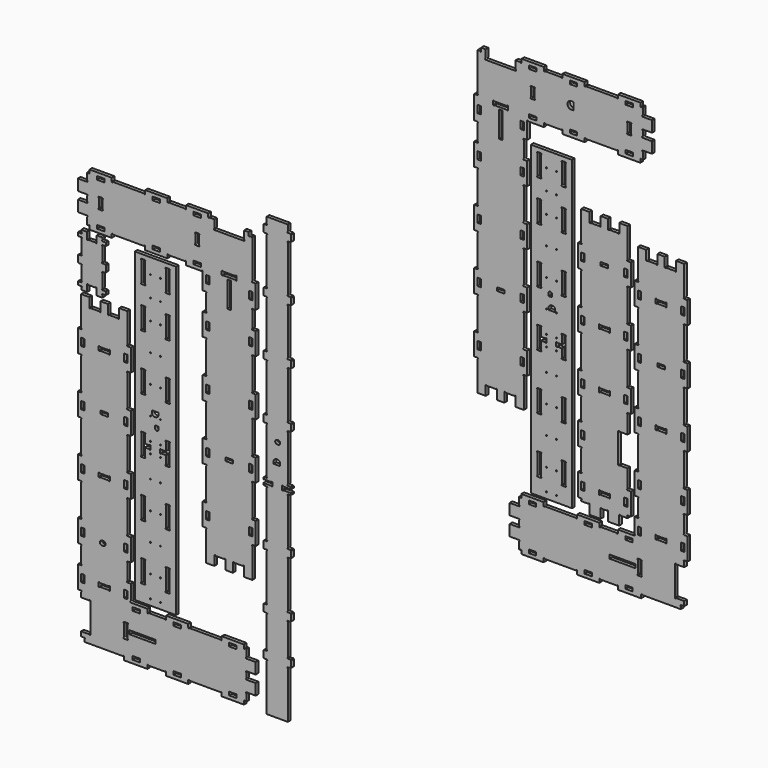
from build123d import *

# Parameters (mm, degrees)
F0_W      = 18
F0_H      = 40
F0_W_2    = 40
F0_H_2    = 18
F0_W_3    = 140
F0_H_3    = 20
F1_DEPTH  = 18
F2_DEPTH  = 18
F3_DEPTH  = 18
F4_DEPTH  = 18
F5_W      = 18
F5_H      = 40
F5_W_2    = 40
F5_H_2    = 18
F5_W_3    = 20
F5_H_3    = 140
F6_DEPTH  = 18
F7_DEPTH  = 18
F5_W_4    = 140
F5_H_4    = 20
F8_DEPTH  = 18
F0_W_4    = 20
F0_H_4    = 140
F9_DEPTH  = 18
F10_DEPTH = 18


# Not quite as in the source:
# - ends of sketch curves that miss each other by under 0.0002 mm in the source are joined


with BuildPart() as f1:
    # F0 (on Front) → F1 (new body)
    with BuildSketch(Plane.XZ):
        with BuildLine():
            Line((183.313294, -1175), (302.813294, -1175))
            Line((302.813294, -1175), (302.813294, -1157.249995))
            ThreePointArc((302.813294, -1157.249995), (305.9533004461, -1153.9924176785), (309.3333033944, -1157.0002460474))
            Line((309.3333033944, -1157.0002460474), (316.117908, -1157.000513))
            Line((316.117908, -1157.000513), (316.117908, -1118.520523))
            ThreePointArc((316.117908, -1118.520523), (313.100645213, -1115.1400374238), (316.3679080001, -1112.0005229167))
            Line((316.3679080001, -1112.0005229167), (366.117908, -1112.000523))
            Line((366.117908, -1112.000523), (366.117908, -1052.500523))
            Line((366.117908, -1052.500523), (316.367908, -1052.500523))
            ThreePointArc((316.367908, -1052.500523), (313.1102104923, -1049.3606421597), (316.1179080369, -1045.9805234706))
            Line((316.1179080369, -1045.9805234706), (316.117908, -1018.520523))
            ThreePointArc((316.117908, -1018.520523), (313.100645213, -1015.1400374238), (316.3679080001, -1012.0005229167))
            Line((316.3679080001, -1012.0005229167), (366.117908, -1012.000523))
            Line((366.117908, -1012.000523), (366.117908, -952.500523))
            Line((366.117908, -952.500523), (316.367908, -952.500523))
            ThreePointArc((316.367908, -952.500523), (313.1102104923, -949.3606421597), (316.1179080369, -945.9805234706))
            Line((316.1179080369, -945.9805234706), (316.117908, -907.500513))
            Line((316.117908, -907.500513), (309.333284, -907.500246))
            ThreePointArc((309.333284, -907.500246), (305.9526828215, -910.5173759685), (302.8132941096, -907.2499950002))
            Line((302.8132941096, -907.2499950002), (302.813294, -889.5))
            Line((302.813294, -889.5), (183.313294, -889.5))
            Line((183.313294, -889.5), (183.313294, -907.25))
            ThreePointArc((183.313294, -907.25), (180.1734131597, -910.5076975077), (176.7932944706, -907.4999999631))
            Line((176.7932944706, -907.4999999631), (9.333294, -907.5))
            ThreePointArc((9.333294, -907.5), (5.9528084238, -910.517262787), (2.8132939167, -907.2499999999))
            Line((2.8132939167, -907.2499999999), (2.813294, -889.5))
            Line((2.813294, -889.5), (-116.686706, -889.5))
            Line((-116.686706, -889.5), (-116.686706, -907.25))
            ThreePointArc((-116.686706, -907.25), (-119.8265868403, -910.5076975077), (-123.2067055294, -907.4999999631))
            Line((-123.2067055294, -907.4999999631), (-210.666706, -907.5))
            ThreePointArc((-210.666706, -907.5), (-214.0471915762, -910.517262787), (-217.1867060833, -907.2499999999))
            Line((-217.1867060833, -907.2499999999), (-217.186706, -889.5))
            Line((-217.186706, -889.5), (-306.702998, -889.5))
            ThreePointArc((-306.702998, -889.5), (-309.9606955077, -886.3601191597), (-306.9529979631, -882.9800004706))
            Line((-306.9529979631, -882.9800004706), (-306.952998, -799.734388))
            Line((-306.952998, -799.734388), (-324.702998, -799.734388))
            ThreePointArc((-324.702998, -799.734388), (-327.9606955077, -796.5945071597), (-324.9529979631, -793.2143884706))
            Line((-324.9529979631, -793.2143884706), (-324.952998, -705.754388))
            ThreePointArc((-324.952998, -705.754388), (-327.970260787, -702.3739024238), (-324.7029979999, -699.2343879167))
            Line((-324.7029979999, -699.2343879167), (-306.952998, -699.234388))
            Line((-306.952998, -699.234388), (-306.952998, -579.734388))
            Line((-306.952998, -579.734388), (-324.702998, -579.734388))
            ThreePointArc((-324.702998, -579.734388), (-327.9606955077, -576.5945071597), (-324.9529979631, -573.2143884706))
            Line((-324.9529979631, -573.2143884706), (-324.952998, -405.754388))
            ThreePointArc((-324.952998, -405.754388), (-327.970260787, -402.3739024238), (-324.7029979999, -399.2343879167))
            Line((-324.7029979999, -399.2343879167), (-306.952998, -399.234388))
            Line((-306.952998, -399.234388), (-306.952998, -279.734388))
            Line((-306.952998, -279.734388), (-324.702998, -279.734388))
            ThreePointArc((-324.702998, -279.734388), (-327.9606955077, -276.5945071597), (-324.9529979631, -273.2143884706))
            Line((-324.9529979631, -273.2143884706), (-324.952998, -105.754388))
            ThreePointArc((-324.952998, -105.754388), (-327.970260787, -102.3739024238), (-324.7029979999, -99.2343879167))
            Line((-324.7029979999, -99.2343879167), (-306.952998, -99.234388))
            Line((-306.952998, -99.234388), (-306.952998, 20.265612))
            Line((-306.952998, 20.265612), (-324.702998, 20.265612))
            ThreePointArc((-324.702998, 20.265612), (-327.9606955077, 23.4054928403), (-324.9529979631, 26.7856115294))
            Line((-324.9529979631, 26.7856115294), (-324.952998, 194.245612))
            ThreePointArc((-324.952998, 194.245612), (-327.970260787, 197.6260975762), (-324.7029979999, 200.7656120833))
            Line((-324.7029979999, 200.7656120833), (-306.952998, 200.765612))
            Line((-306.952998, 200.765612), (-306.952998, 320.265612))
            Line((-306.952998, 320.265612), (-324.702998, 320.265612))
            ThreePointArc((-324.702998, 320.265612), (-327.9606955077, 323.4054928403), (-324.9529979631, 326.7856115294))
            Line((-324.9529979631, 326.7856115294), (-324.952998, 486.960693))
            Line((-324.952998, 486.960693), (-369.452998, 486.960693))
            Line((-369.452998, 486.960693), (-369.452998, 437.210693))
            ThreePointArc((-369.452998, 437.210693), (-372.5928788403, 433.9529954923), (-375.9729975294, 436.9606930369))
            Line((-375.9729975294, 436.9606930369), (-423.432998, 436.960693))
            ThreePointArc((-423.432998, 436.960693), (-426.8134835762, 433.943430213), (-429.9529980833, 437.2106930001))
            Line((-429.9529980833, 437.2106930001), (-429.952998, 486.960693))
            Line((-429.952998, 486.960693), (-469.452998, 486.960693))
            Line((-469.452998, 486.960693), (-469.452998, 437.210693))
            ThreePointArc((-469.452998, 437.210693), (-472.5928788403, 433.9529954923), (-475.9729975294, 436.9606930369))
            Line((-475.9729975294, 436.9606930369), (-523.432998, 436.960693))
            ThreePointArc((-523.432998, 436.960693), (-526.8134835762, 433.943430213), (-529.9529980833, 437.2106930001))
            Line((-529.9529980833, 437.2106930001), (-529.952998, 486.960693))
            Line((-529.952998, 486.960693), (-574.452998, 486.960693))
            Line((-574.452998, 486.960693), (-574.452998, 326.785612))
            ThreePointArc((-574.452998, 326.785612), (-571.435735213, 323.4051264238), (-574.7029980001, 320.2656119167))
            Line((-574.7029980001, 320.2656119167), (-592.452998, 320.265612))
            Line((-592.452998, 320.265612), (-592.452998, 200.765612))
            Line((-592.452998, 200.765612), (-574.702998, 200.765612))
            ThreePointArc((-574.702998, 200.765612), (-571.4453004923, 197.6257311597), (-574.4529980369, 194.2456124706))
            Line((-574.4529980369, 194.2456124706), (-574.452998, 26.785612))
            ThreePointArc((-574.452998, 26.785612), (-571.435735213, 23.4051264238), (-574.7029980001, 20.2656119167))
            Line((-574.7029980001, 20.2656119167), (-592.452998, 20.265612))
            Line((-592.452998, 20.265612), (-592.452998, -99.234388))
            Line((-592.452998, -99.234388), (-574.702998, -99.234388))
            ThreePointArc((-574.702998, -99.234388), (-571.4453004923, -102.3742688403), (-574.4529980369, -105.7543875294))
            Line((-574.4529980369, -105.7543875294), (-574.452998, -273.214388))
            ThreePointArc((-574.452998, -273.214388), (-571.435735213, -276.5948735762), (-574.7029980001, -279.7343880833))
            Line((-574.7029980001, -279.7343880833), (-592.452998, -279.734388))
            Line((-592.452998, -279.734388), (-592.452998, -399.234388))
            Line((-592.452998, -399.234388), (-574.702998, -399.234388))
            ThreePointArc((-574.702998, -399.234388), (-571.4453004923, -402.3742688403), (-574.4529980369, -405.7543875294))
            Line((-574.4529980369, -405.7543875294), (-574.452998, -573.214388))
            ThreePointArc((-574.452998, -573.214388), (-571.435735213, -576.5948735762), (-574.7029980001, -579.7343880833))
            Line((-574.7029980001, -579.7343880833), (-592.452998, -579.734388))
            Line((-592.452998, -579.734388), (-592.452998, -699.234388))
            Line((-592.452998, -699.234388), (-574.702998, -699.234388))
            ThreePointArc((-574.702998, -699.234388), (-571.4453004923, -702.3742688403), (-574.4529980369, -705.7543875294))
            Line((-574.4529980369, -705.7543875294), (-574.452998, -793.214388))
            ThreePointArc((-574.452998, -793.214388), (-571.435735213, -796.5948735762), (-574.7029980001, -799.7343880833))
            Line((-574.7029980001, -799.7343880833), (-592.452998, -799.734388))
            Line((-592.452998, -799.734388), (-592.452998, -919.234388))
            Line((-592.452998, -919.234388), (-574.702998, -919.234388))
            ThreePointArc((-574.702998, -919.234388), (-571.4453004923, -922.3742688403), (-574.4529980369, -925.7543875294))
            Line((-574.4529980369, -925.7543875294), (-574.452998, -952.000316))
            Line((-574.452998, -952.000316), (-530.972998, -952.000316))
            ThreePointArc((-530.972998, -952.000316), (-527.5925124238, -948.983053213), (-524.4529979167, -952.2503160001))
            Line((-524.4529979167, -952.2503160001), (-524.452998, -1112.250316))
            ThreePointArc((-524.452998, -1112.250316), (-527.5928788403, -1115.5080135077), (-530.9729975294, -1112.5003159631))
            Line((-530.9729975294, -1112.5003159631), (-574.452998, -1112.500316))
            Line((-574.452998, -1112.500316), (-574.452998, -1137.000316))
            Line((-574.452998, -1137.000316), (-556.702998, -1137.000316))
            ThreePointArc((-556.702998, -1137.000316), (-553.4453004923, -1140.1401968403), (-556.4529980369, -1143.5203155294))
            Line((-556.4529980369, -1143.5203155294), (-556.452998, -1157.000315))
            Line((-556.452998, -1157.000315), (-348.977728, -1157.000009))
            ThreePointArc((-348.977728, -1157.000009), (-345.5972459509, -1153.9827410395), (-342.4577269106, -1157.2500000001))
            Line((-342.4577269106, -1157.2500000001), (-342.457727, -1175))
            Line((-342.457727, -1175), (-217.186706, -1175))
            Line((-217.186706, -1175), (-217.186706, -1157.25))
            ThreePointArc((-217.186706, -1157.25), (-214.0468251597, -1153.9923024923), (-210.6667064706, -1157.0000000369))
            Line((-210.6667064706, -1157.0000000369), (-123.206706, -1157))
            ThreePointArc((-123.206706, -1157), (-119.8262204238, -1153.9827372131), (-116.6867059167, -1157.2500000001))
            Line((-116.6867059167, -1157.2500000001), (-116.686706, -1175))
            Line((-116.686706, -1175), (2.813294, -1175))
            Line((2.813294, -1175), (2.813294, -1157.25))
            ThreePointArc((2.813294, -1157.25), (5.9531748403, -1153.9923024923), (9.3332935294, -1157.0000000369))
            Line((9.3332935294, -1157.0000000369), (176.793294, -1157))
            ThreePointArc((176.793294, -1157), (180.1737795762, -1153.9827372131), (183.3132940833, -1157.2500000001))
            Line((183.3132940833, -1157.2500000001), (183.313294, -1175))
        make_face()
        with BuildLine():
            ThreePointArc((-342.9529979891, -998.5178928555), (-345.9678398614, -995.1386665833), (-342.7029979991, -992.0003152124))
            Line((-342.7029979991, -992.0003152124), (-324.702998, -992.000316))
            ThreePointArc((-324.702998, -992.000316), (-321.4453073491, -995.1389416301), (-324.4529979547, -998.5178935807))
            Line((-324.4529979547, -998.5178935807), (-324.452998, -1065.982739))
            ThreePointArc((-324.452998, -1065.982739), (-321.4381561386, -1069.3619654167), (-324.7029980009, -1072.5003167876))
            Line((-324.7029980009, -1072.5003167876), (-342.702998, -1072.500316))
            ThreePointArc((-342.702998, -1072.500316), (-345.9606886509, -1069.3616903699), (-342.9529980453, -1065.9827384193))
            Line((-342.9529980453, -1065.9827384193), (-342.9529979891, -998.5178928555))
        make_face(mode=Mode.SUBTRACT)
        with Locations((-565.702998, -859.484388)):
            Rectangle(F0_W, F0_H, mode=Mode.SUBTRACT)
        with Locations((-565.702998, -639.484388)):
            Rectangle(F0_W, F0_H, mode=Mode.SUBTRACT)
        Polygon((-473.524462, -658.100617), (-473.551633, -657.552381), (-473.551323, -657.237725), (-473.542932, -656.923857), (-473.526522, -656.610923), (-473.502154, -656.299068), (-473.469886, -655.98844), (-473.429781, -655.679185), (-473.381899, -655.37145), (-473.326299, -655.065381), (-473.263044, -654.761124), (-473.192193, -654.458826), (-473.113806, -654.158634), (-473.027945, -653.860693), (-472.93467, -653.565151), (-472.834042, -653.272154), (-472.72612, -652.981848), (-472.610966, -652.694381), (-472.48864, -652.409897), (-472.359203, -652.128545), (-472.222715, -651.850469), (-472.079237, -651.575818), (-471.928829, -651.304737), (-471.771552, -651.037373), (-471.607466, -650.773872), (-471.436633, -650.514381), (-471.259112, -650.259046), (-471.074964, -650.008013), (-470.884249, -649.76143), (-470.687029, -649.519443), (-470.483363, -649.282198), (-470.273312, -649.049842), (-470.056938, -648.82252), (-469.834299, -648.600381), (-469.549184, -648.322479), (-469.257469, -648.052825), (-468.959351, -647.791495), (-468.655029, -647.538563), (-468.344698, -647.294106), (-468.028557, -647.058199), (-467.706803, -646.830918), (-467.379633, -646.612339), (-467.047244, -646.402537), (-466.709833, -646.201588), (-466.367599, -646.009568), (-466.020737, -645.826553), (-465.669446, -645.652617), (-465.313922, -645.487837), (-464.954363, -645.332289), (-464.590966, -645.186047), (-464.223929, -645.049189), (-463.853448, -644.921789), (-463.479721, -644.803923), (-463.102945, -644.695667), (-462.723318, -644.597097), (-462.341036, -644.508288), (-461.956298, -644.429315), (-461.569299, -644.360256), (-461.180239, -644.301184), (-460.789312, -644.252177), (-460.396718, -644.213309), (-460.002654, -644.184657), (-459.607315, -644.166295), (-459.210901, -644.158301), (-458.813608, -644.160748), (-458.415633, -644.173714), (-457.989627, -644.158147), (-457.564239, -644.1534), (-457.139667, -644.159401), (-456.716107, -644.176079), (-456.293756, -644.203362), (-455.872811, -644.241179), (-455.453468, -644.289459), (-455.035924, -644.348131), (-454.620377, -644.417123), (-454.207023, -644.496364), (-453.796058, -644.585782), (-453.38768, -644.685308), (-452.982085, -644.794868), (-452.579469, -644.914392), (-452.180031, -645.043809), (-451.783966, -645.183047), (-451.391472, -645.332035), (-451.002744, -645.490702), (-450.617981, -645.658976), (-450.237378, -645.836787), (-449.861132, -646.024062), (-449.489441, -646.220731), (-449.1225, -646.426722), (-448.760508, -646.641964), (-448.40366, -646.866386), (-448.052153, -647.099916), (-447.706184, -647.342483), (-447.36595, -647.594016), (-447.031648, -647.854444), (-446.703475, -648.123694), (-446.381626, -648.401697), (-446.066299, -648.688381), (-445.671937, -649.082422), (-445.300148, -649.494834), (-444.951383, -649.924551), (-444.626091, -650.370506), (-444.324721, -650.831633), (-444.047721, -651.306865), (-443.795542, -651.795136), (-443.568633, -652.295381), (-443.367442, -652.806531), (-443.192419, -653.327521), (-443.044014, -653.857285), (-442.922674, -654.394756), (-442.828851, -654.938867), (-442.762992, -655.488553), (-442.725548, -656.042746), (-442.716966, -656.600381), (-442.721229, -656.913755), (-442.733479, -657.226281), (-442.753655, -657.537814), (-442.781695, -657.848209), (-442.817541, -658.15732), (-442.86113, -658.465004), (-442.912403, -658.771114), (-442.971299, -659.075506), (-443.037758, -659.378034), (-443.111719, -659.678554), (-443.193121, -659.976921), (-443.281904, -660.27299), (-443.378007, -660.566615), (-443.48137, -660.857652), (-443.591932, -661.145956), (-443.709633, -661.431381), (-443.834412, -661.713782), (-443.966208, -661.993015), (-444.104962, -662.268935), (-444.250612, -662.541396), (-444.403098, -662.810254), (-444.562359, -663.075363), (-444.728336, -663.336579), (-444.900966, -663.593756), (-445.08019, -663.846749), (-445.265948, -664.095414), (-445.458178, -664.339605), (-445.65682, -664.579178), (-445.861814, -664.813986), (-446.073099, -665.043886), (-446.290614, -665.268733), (-446.514299, -665.488381), (-446.814824, -665.753096), (-447.121277, -666.0097), (-447.433479, -666.258125), (-447.751247, -666.498308), (-448.074403, -666.730182), (-448.402764, -666.953681), (-448.736151, -667.168742), (-449.074383, -667.375297), (-449.417278, -667.573282), (-449.764658, -667.762632), (-450.116339, -667.94328), (-450.472143, -668.115162), (-450.831888, -668.278212), (-451.195395, -668.432364), (-451.562481, -668.577553), (-451.932966, -668.713714), (-452.30667, -668.840781), (-452.683413, -668.958689), (-453.063013, -669.067373), (-453.445289, -669.166766), (-453.830062, -669.256804), (-454.21715, -669.337421), (-454.606373, -669.408552), (-454.997549, -669.470131), (-455.3905, -669.522092), (-455.785043, -669.564372), (-456.180998, -669.596903), (-456.4282935464, -669.611047), (-456.578185, -669.61962), (-456.976422, -669.632459), (-457.37553, -669.635353), (-457.775327, -669.628238), (-458.175633, -669.611047), (-458.58489, -669.626762), (-458.993534, -669.631955), (-459.401373, -669.626696), (-459.808216, -669.611058), (-460.213872, -669.585111), (-460.618148, -669.548926), (-461.020855, -669.502576), (-461.421799, -669.446131), (-461.820791, -669.379662), (-462.217638, -669.303241), (-462.612149, -669.21694), (-463.004133, -669.120829), (-463.393398, -669.014979), (-463.779753, -668.899463), (-464.163006, -668.774351), (-464.542966, -668.639714), (-464.919442, -668.495624), (-465.292242, -668.342153), (-465.661175, -668.179371), (-466.026049, -668.007349), (-466.386674, -667.82616), (-466.742857, -667.635874), (-467.094407, -667.436563), (-467.441133, -667.228297), (-467.782843, -667.011149), (-468.119346, -666.785189), (-468.450451, -666.550489), (-468.775966, -666.30712), (-469.0957, -666.055154), (-469.409461, -665.794661), (-469.717058, -665.525713), (-470.018299, -665.248381), (-470.416252, -664.870301), (-470.792794, -664.47374), (-471.147454, -664.059719), (-471.479758, -663.629256), (-471.789234, -663.183371), (-472.075409, -662.723084), (-472.337811, -662.249414), (-472.575966, -661.763381), (-472.789403, -661.266004), (-472.977648, -660.758303), (-473.14023, -660.241297), (-473.276674, -659.716006), (-473.38651, -659.183449), (-473.469263, -658.644646), align=None, mode=Mode.SUBTRACT)
        with BuildLine():
            ThreePointArc((-425.9705748555, -850.2343880109), (-422.5913485833, -847.2195461386), (-419.4529972124, -850.4843880009))
            Line((-419.4529972124, -850.4843880009), (-419.452998, -868.484388))
            ThreePointArc((-419.452998, -868.484388), (-422.5916236301, -871.7420786509), (-425.9705755807, -868.7343880453))
            Line((-425.9705755807, -868.7343880453), (-473.435421, -868.734388))
            ThreePointArc((-473.435421, -868.734388), (-476.8146474167, -871.7492298614), (-479.9529987876, -868.4843879991))
            Line((-479.9529987876, -868.4843879991), (-479.952998, -850.484388))
            ThreePointArc((-479.952998, -850.484388), (-476.8143723699, -847.2266973491), (-473.4354204193, -850.2343879547))
            Line((-473.4354204193, -850.2343879547), (-425.9705748555, -850.2343880109))
        make_face(mode=Mode.SUBTRACT)
        with Locations((-333.702998, -859.484388)):
            Rectangle(F0_W, F0_H, mode=Mode.SUBTRACT)
        with Locations((-333.702998, -639.484388)):
            Rectangle(F0_W, F0_H, mode=Mode.SUBTRACT)
        with Locations((-276.936706, -1148.25)):
            Rectangle(F0_W_2, F0_H_2, mode=Mode.SUBTRACT)
        with Locations((-242.702998, -1032.250316)):
            Rectangle(F0_W_3, F0_H_3, mode=Mode.SUBTRACT)
        with Locations((-276.936706, -916.25)):
            Rectangle(F0_W_2, F0_H_2, mode=Mode.SUBTRACT)
        with Locations((-56.936706, -1148.25)):
            Rectangle(F0_W_2, F0_H_2, mode=Mode.SUBTRACT)
        with Locations((-56.936706, -916.25)):
            Rectangle(F0_W_2, F0_H_2, mode=Mode.SUBTRACT)
        with Locations((-565.702998, -339.484388)):
            Rectangle(F0_W, F0_H, mode=Mode.SUBTRACT)
        with BuildLine():
            ThreePointArc((-425.9705748555, -330.2343880109), (-422.5913485833, -327.2195461386), (-419.4529972124, -330.4843880009))
            Line((-419.4529972124, -330.4843880009), (-419.452998, -348.484388))
            ThreePointArc((-419.452998, -348.484388), (-422.5916236301, -351.7420786509), (-425.9705755807, -348.7343880453))
            Line((-425.9705755807, -348.7343880453), (-473.435421, -348.734388))
            ThreePointArc((-473.435421, -348.734388), (-476.8146474167, -351.7492298614), (-479.9529987876, -348.4843879991))
            Line((-479.9529987876, -348.4843879991), (-479.952998, -330.484388))
            ThreePointArc((-479.952998, -330.484388), (-476.8143723699, -327.2266973491), (-473.4354204193, -330.2343879547))
            Line((-473.4354204193, -330.2343879547), (-425.9705748555, -330.2343880109))
        make_face(mode=Mode.SUBTRACT)
        with Locations((-333.702998, -339.484388)):
            Rectangle(F0_W, F0_H, mode=Mode.SUBTRACT)
        with Locations((-565.702998, -39.484388)):
            Rectangle(F0_W, F0_H, mode=Mode.SUBTRACT)
        with Locations((-449.702998, -39.484388)):
            Rectangle(F0_W_2, F0_H_2, mode=Mode.SUBTRACT)
        with Locations((-333.702998, -39.484388)):
            Rectangle(F0_W, F0_H, mode=Mode.SUBTRACT)
        with Locations((243.063294, -1148.25)):
            Rectangle(F0_W_2, F0_H_2, mode=Mode.SUBTRACT)
        with Locations((243.063294, -916.25)):
            Rectangle(F0_W_2, F0_H_2, mode=Mode.SUBTRACT)
        with Locations((-565.702998, 260.515612)):
            Rectangle(F0_W, F0_H, mode=Mode.SUBTRACT)
        with BuildLine():
            ThreePointArc((-425.9705748555, 269.7656119891), (-422.5913485833, 272.7804538614), (-419.4529972124, 269.5156119991))
            Line((-419.4529972124, 269.5156119991), (-419.452998, 251.515612))
            ThreePointArc((-419.452998, 251.515612), (-422.5916236301, 248.2579213491), (-425.9705755807, 251.2656119547))
            Line((-425.9705755807, 251.2656119547), (-473.435421, 251.265612))
            ThreePointArc((-473.435421, 251.265612), (-476.8146474167, 248.2507701386), (-479.9529987876, 251.5156120009))
            Line((-479.9529987876, 251.5156120009), (-479.952998, 269.515612))
            ThreePointArc((-479.952998, 269.515612), (-476.8143723699, 272.7733026509), (-473.4354204193, 269.7656120453))
            Line((-473.4354204193, 269.7656120453), (-425.9705748555, 269.7656119891))
        make_face(mode=Mode.SUBTRACT)
        with Locations((-333.702998, 260.515612)):
            Rectangle(F0_W, F0_H, mode=Mode.SUBTRACT)
    extrude(amount=F1_DEPTH)


with BuildPart() as f2:
    # F0 (on Front) → F2 (new body)
    with BuildSketch(Plane.XZ):
        with BuildLine():
            Line((-591.564675, 632.919501), (-588.564672, 629.919498))
            Line((-588.564672, 629.919498), (-573.564657, 629.919498))
            ThreePointArc((-573.564657, 629.919498), (-570.554657, 626.909498), (-573.564657, 623.899498))
            Line((-573.564657, 623.899498), (-573.564657, 548.938173))
            ThreePointArc((-573.564657, 548.938173), (-570.554657, 545.928173), (-573.564657, 542.918173))
            Line((-573.564657, 542.918173), (-591.564974, 542.918173))
            Line((-591.564974, 542.918173), (-591.564974, 524.918282))
            Line((-591.564974, 524.918282), (-573.564657, 524.918282))
            ThreePointArc((-573.564657, 524.918282), (-570.554657, 521.908282), (-573.564657, 518.898282))
            Line((-573.564657, 518.898282), (-573.564657, 506.918264))
            Line((-573.564657, 506.918264), (-542.564626, 506.918264))
            Line((-542.564626, 506.918264), (-542.564626, 542.918173))
            ThreePointArc((-542.564626, 542.918173), (-539.554626, 545.928173), (-536.544626, 542.918173))
            Line((-536.544626, 542.918173), (-496.585606, 542.918173))
            ThreePointArc((-496.585606, 542.918173), (-493.575606, 545.928173), (-490.565606, 542.918173))
            Line((-490.565606, 542.918173), (-490.565606, 506.918264))
            Line((-490.565606, 506.918264), (-459.565575, 506.918264))
            Line((-459.565575, 506.918264), (-459.565575, 518.898282))
            ThreePointArc((-459.565575, 518.898282), (-462.575575, 521.908282), (-459.565575, 524.918282))
            Line((-459.565575, 524.918282), (-441.565258, 524.918282))
            Line((-441.565258, 524.918282), (-441.565258, 542.918173))
            Line((-441.565258, 542.918173), (-459.565575, 542.918173))
            ThreePointArc((-459.565575, 542.918173), (-462.575575, 545.928173), (-459.565575, 548.938173))
            Line((-459.565575, 548.938173), (-459.565575, 623.899498))
            ThreePointArc((-459.565575, 623.899498), (-462.575575, 626.909498), (-459.565575, 629.919498))
            Line((-459.565575, 629.919498), (-444.56556, 629.919498))
            Line((-444.56556, 629.919498), (-441.565557, 632.919501))
            Line((-441.565557, 632.919501), (-441.565557, 666.919535))
            Line((-441.565557, 666.919535), (-444.56556, 669.919538))
            Line((-444.56556, 669.919538), (-459.565575, 669.919538))
            ThreePointArc((-459.565575, 669.919538), (-462.575575, 672.929538), (-459.565575, 675.939538))
            Line((-459.565575, 675.939538), (-459.565575, 750.898514))
            ThreePointArc((-459.565575, 750.898514), (-462.575575, 753.908514), (-459.565575, 756.918514))
            Line((-459.565575, 756.918514), (-441.565557, 756.918514))
            Line((-441.565557, 756.918514), (-441.565557, 774.918405))
            Line((-441.565557, 774.918405), (-459.565575, 774.918405))
            ThreePointArc((-459.565575, 774.918405), (-462.575575, 777.928405), (-459.565575, 780.938405))
            Line((-459.565575, 780.938405), (-459.565575, 792.918413))
            Line((-459.565575, 792.918413), (-490.565606, 792.918413))
            Line((-490.565606, 792.918413), (-490.565606, 756.962246))
            ThreePointArc((-490.565606, 756.962246), (-493.575606, 753.952246), (-496.585606, 756.962246))
            Line((-496.585606, 756.962246), (-536.544626, 756.962246))
            ThreePointArc((-536.544626, 756.962246), (-539.554626, 753.952246), (-542.564626, 756.962246))
            Line((-542.564626, 756.962246), (-542.564626, 792.918413))
            Line((-542.564626, 792.918413), (-573.564657, 792.918413))
            Line((-573.564657, 792.918413), (-573.564657, 780.938405))
            ThreePointArc((-573.564657, 780.938405), (-570.554657, 777.928405), (-573.564657, 774.918405))
            Line((-573.564657, 774.918405), (-591.564675, 774.918405))
            Line((-591.564675, 774.918405), (-591.564675, 756.918514))
            Line((-591.564675, 756.918514), (-573.564657, 756.918514))
            ThreePointArc((-573.564657, 756.918514), (-570.554657, 753.908514), (-573.564657, 750.898514))
            Line((-573.564657, 750.898514), (-573.564657, 675.939538))
            ThreePointArc((-573.564657, 675.939538), (-570.554657, 672.929538), (-573.564657, 669.919538))
            Line((-573.564657, 669.919538), (-588.564672, 669.919538))
            Line((-588.564672, 669.919538), (-591.564675, 666.919535))
            Line((-591.564675, 666.919535), (-591.564675, 632.919501))
        make_face()
    extrude(amount=F2_DEPTH)


with BuildPart() as f3:
    # F0 (on Front) → F3 (new body)
    with BuildSketch(Plane.XZ):
        Polygon((-285.358585, -869.5), (-63.26891, -869.5), (-63.26891, 783.266038), (-285.358584, 783.266038), align=None)
        with BuildLine():
            ThreePointArc((-201.358517, -833.60319), (-199.2371966564, -834.4818696564), (-198.358517, -836.60319))
            ThreePointArc((-198.358517, -836.60319), (-199.2371966564, -838.7245103436), (-201.358517, -839.60319))
            ThreePointArc((-201.358517, -839.60319), (-203.4798373436, -838.7245103436), (-204.358517, -836.60319))
            ThreePointArc((-204.358517, -836.60319), (-203.4798373436, -834.4818696564), (-201.358517, -833.60319))
        make_face(mode=Mode.SUBTRACT)
        with BuildLine():
            Line((-249.608535, -773.731149), (-249.608535, -665.271029))
            ThreePointArc((-249.608535, -665.271029), (-252.618535, -662.261029), (-249.608535, -659.251029))
            Line((-249.608535, -659.251029), (-231.108517, -659.251029))
            ThreePointArc((-231.108517, -659.251029), (-228.098517, -662.261029), (-231.108517, -665.271029))
            Line((-231.108517, -665.271029), (-231.108517, -773.731149))
            ThreePointArc((-231.108517, -773.731149), (-228.098517, -776.741149), (-231.108517, -779.751149))
            Line((-231.108517, -779.751149), (-249.608535, -779.751149))
            ThreePointArc((-249.608535, -779.751149), (-252.618535, -776.741149), (-249.608535, -773.731149))
        make_face(mode=Mode.SUBTRACT)
        with BuildLine():
            ThreePointArc((-201.358517, -716.49985), (-199.2371966564, -717.3785296564), (-198.358517, -719.49985))
            ThreePointArc((-198.358517, -719.49985), (-199.2371966564, -721.6211703436), (-201.358517, -722.49985))
            ThreePointArc((-201.358517, -722.49985), (-203.4798373436, -721.6211703436), (-204.358517, -719.49985))
            ThreePointArc((-204.358517, -719.49985), (-203.4798373436, -717.3785296564), (-201.358517, -716.49985))
        make_face(mode=Mode.SUBTRACT)
        with BuildLine():
            ThreePointArc((-147.268942, -833.60319), (-145.1476216564, -834.4818696564), (-144.268942, -836.60319))
            ThreePointArc((-144.268942, -836.60319), (-145.1476216564, -838.7245103436), (-147.268942, -839.60319))
            ThreePointArc((-147.268942, -839.60319), (-149.3902623436, -838.7245103436), (-150.268942, -836.60319))
            ThreePointArc((-150.268942, -836.60319), (-149.3902623436, -834.4818696564), (-147.268942, -833.60319))
        make_face(mode=Mode.SUBTRACT)
        with BuildLine():
            ThreePointArc((-147.268942, -716.49985), (-145.1476216564, -717.3785296564), (-144.268942, -719.49985))
            ThreePointArc((-144.268942, -719.49985), (-145.1476216564, -721.6211703436), (-147.268942, -722.49985))
            ThreePointArc((-147.268942, -722.49985), (-149.3902623436, -721.6211703436), (-150.268942, -719.49985))
            ThreePointArc((-150.268942, -719.49985), (-149.3902623436, -717.3785296564), (-147.268942, -716.49985))
        make_face(mode=Mode.SUBTRACT)
        with BuildLine():
            Line((-99.018924, -665.26979), (-99.018924, -773.72991))
            ThreePointArc((-99.018924, -773.72991), (-96.008924, -776.73991), (-99.018924, -779.74991))
            Line((-99.018924, -779.74991), (-117.518942, -779.74991))
            ThreePointArc((-117.518942, -779.74991), (-120.528942, -776.73991), (-117.518942, -773.72991))
            Line((-117.518942, -773.72991), (-117.518942, -665.26979))
            ThreePointArc((-117.518942, -665.26979), (-120.528942, -662.25979), (-117.518942, -659.24979))
            Line((-117.518942, -659.24979), (-99.018924, -659.24979))
            ThreePointArc((-99.018924, -659.24979), (-96.008924, -662.25979), (-99.018924, -665.26979))
        make_face(mode=Mode.SUBTRACT)
        with BuildLine():
            ThreePointArc((-201.358517, -566.49985), (-199.2371966564, -567.3785296564), (-198.358517, -569.49985))
            ThreePointArc((-198.358517, -569.49985), (-199.2371966564, -571.6211703436), (-201.358517, -572.49985))
            ThreePointArc((-201.358517, -572.49985), (-203.4798373436, -571.6211703436), (-204.358517, -569.49985))
            ThreePointArc((-204.358517, -569.49985), (-203.4798373436, -567.3785296564), (-201.358517, -566.49985))
        make_face(mode=Mode.SUBTRACT)
        with BuildLine():
            Line((-231.108517, -479.750849), (-249.608535, -479.750849))
            ThreePointArc((-249.608535, -479.750849), (-252.618535, -476.740849), (-249.608535, -473.730849))
            Line((-249.608535, -473.730849), (-249.608535, -365.270729))
            ThreePointArc((-249.608535, -365.270729), (-252.618535, -362.260729), (-249.608535, -359.250729))
            Line((-249.608535, -359.250729), (-231.108517, -359.250729))
            ThreePointArc((-231.108517, -359.250729), (-228.098517, -362.260729), (-231.108517, -365.270729))
            Line((-231.108517, -365.270729), (-231.108517, -473.730849))
            ThreePointArc((-231.108517, -473.730849), (-228.098517, -476.740849), (-231.108517, -479.750849))
        make_face(mode=Mode.SUBTRACT)
        with BuildLine():
            ThreePointArc((-201.358517, -416.49985), (-199.2371966564, -417.3785296564), (-198.358517, -419.49985))
            ThreePointArc((-198.358517, -419.49985), (-199.2371966564, -421.6211703436), (-201.358517, -422.49985))
            ThreePointArc((-201.358517, -422.49985), (-203.4798373436, -421.6211703436), (-204.358517, -419.49985))
            ThreePointArc((-204.358517, -419.49985), (-203.4798373436, -417.3785296564), (-201.358517, -416.49985))
        make_face(mode=Mode.SUBTRACT)
        with BuildLine():
            ThreePointArc((-147.268942, -566.49985), (-145.1476216564, -567.3785296564), (-144.268942, -569.49985))
            ThreePointArc((-144.268942, -569.49985), (-145.1476216564, -571.6211703436), (-147.268942, -572.49985))
            ThreePointArc((-147.268942, -572.49985), (-149.3902623436, -571.6211703436), (-150.268942, -569.49985))
            ThreePointArc((-150.268942, -569.49985), (-149.3902623436, -567.3785296564), (-147.268942, -566.49985))
        make_face(mode=Mode.SUBTRACT)
        with BuildLine():
            ThreePointArc((-147.268942, -416.49985), (-145.1476216564, -417.3785296564), (-144.268942, -419.49985))
            ThreePointArc((-144.268942, -419.49985), (-145.1476216564, -421.6211703436), (-147.268942, -422.49985))
            ThreePointArc((-147.268942, -422.49985), (-149.3902623436, -421.6211703436), (-150.268942, -419.49985))
            ThreePointArc((-150.268942, -419.49985), (-149.3902623436, -417.3785296564), (-147.268942, -416.49985))
        make_face(mode=Mode.SUBTRACT)
        with BuildLine():
            Line((-117.518942, -473.72961), (-117.518942, -365.26949))
            ThreePointArc((-117.518942, -365.26949), (-120.528942, -362.25949), (-117.518942, -359.24949))
            Line((-117.518942, -359.24949), (-99.018924, -359.24949))
            ThreePointArc((-99.018924, -359.24949), (-96.008924, -362.25949), (-99.018924, -365.26949))
            Line((-99.018924, -365.26949), (-99.018924, -473.72961))
            ThreePointArc((-99.018924, -473.72961), (-96.008924, -476.73961), (-99.018924, -479.74961))
            Line((-99.018924, -479.74961), (-117.518942, -479.74961))
            ThreePointArc((-117.518942, -479.74961), (-120.528942, -476.73961), (-117.518942, -473.72961))
        make_face(mode=Mode.SUBTRACT)
        with BuildLine():
            ThreePointArc((-201.358517, -266.49985), (-199.2371966564, -267.3785296564), (-198.358517, -269.49985))
            ThreePointArc((-198.358517, -269.49985), (-199.2371966564, -271.6211703436), (-201.358517, -272.49985))
            ThreePointArc((-201.358517, -272.49985), (-203.4798373436, -271.6211703436), (-204.358517, -269.49985))
            ThreePointArc((-204.358517, -269.49985), (-203.4798373436, -267.3785296564), (-201.358517, -266.49985))
        make_face(mode=Mode.SUBTRACT)
        with BuildLine():
            Line((-249.608535, -173.730549), (-249.608535, -65.270429))
            ThreePointArc((-249.608535, -65.270429), (-252.618535, -62.260429), (-249.608535, -59.250429))
            Line((-249.608535, -59.250429), (-231.108525, -59.250429))
            ThreePointArc((-231.108525, -59.2504290016), (-228.0984270016, -62.260331), (-231.108329, -65.2704289984))
            Line((-231.108329, -65.270429), (-231.106868, -110.251463))
            Line((-231.106868, -110.251463), (-206.126829, -110.251463))
            ThreePointArc((-206.126829, -110.251463), (-203.116829, -107.241463), (-200.106829, -110.251463))
            Line((-200.106829, -110.251463), (-200.106829, -128.751481))
            ThreePointArc((-200.106829, -128.751481), (-203.116829, -131.761481), (-206.126829, -128.751481))
            Line((-206.126829, -128.751481), (-231.106868, -128.751481))
            Line((-231.106868, -128.751481), (-231.108329, -173.730549))
            ThreePointArc((-231.108329, -173.7305490016), (-228.0984270016, -176.740647), (-231.108525, -179.7505489984))
            Line((-231.108525, -179.750549), (-249.608535, -179.750549))
            ThreePointArc((-249.608535, -179.750549), (-252.618535, -176.740549), (-249.608535, -173.730549))
        make_face(mode=Mode.SUBTRACT)
        with BuildLine():
            ThreePointArc((-201.358517, -146.503093), (-199.2371966564, -147.3817726564), (-198.358517, -149.503093))
            ThreePointArc((-198.358517, -149.503093), (-199.2371966564, -151.6244133436), (-201.358517, -152.503093))
            ThreePointArc((-201.358517, -152.503093), (-203.4798373436, -151.6244133436), (-204.358517, -149.503093))
            ThreePointArc((-204.358517, -149.503093), (-203.4798373436, -147.3817726564), (-201.358517, -146.503093))
        make_face(mode=Mode.SUBTRACT)
        with BuildLine():
            ThreePointArc((-201.358517, -86.49985), (-199.2371966564, -87.3785296564), (-198.358517, -89.49985))
            ThreePointArc((-198.358517, -89.49985), (-199.2371966564, -91.6211703436), (-201.358517, -92.49985))
            ThreePointArc((-201.358517, -92.49985), (-203.4798373436, -91.6211703436), (-204.358517, -89.49985))
            ThreePointArc((-204.358517, -89.49985), (-203.4798373436, -87.3785296564), (-201.358517, -86.49985))
        make_face(mode=Mode.SUBTRACT)
        Polygon((-175.457354, -20.994449), (-175.457354, -5.631783), (-157.98302, -5.631783), (-157.98302, -20.994449), (-157.985998, -21.427028), (-158.01133, -21.857094), (-158.058674, -22.283832), (-158.127687, -22.706423), (-158.218028, -23.124052), (-158.329356, -23.5359), (-158.461329, -23.941152), (-158.613604, -24.338991), (-158.78584, -24.728599), (-158.977695, -25.10916), (-159.188827, -25.479856), (-159.418895, -25.839871), (-159.667557, -26.188388), (-159.934471, -26.524591), (-160.219295, -26.847661), (-160.521687, -27.156783), (-160.829256, -27.454667), (-161.15032, -27.735604), (-161.484098, -27.999274), (-161.829812, -28.245355), (-162.186682, -28.473527), (-162.553929, -28.683466), (-162.930774, -28.874853), (-163.316437, -29.047366), (-163.710139, -29.200683), (-164.111101, -29.334484), (-164.518543, -29.448447), (-164.931687, -29.542251), (-165.349752, -29.615575), (-165.77196, -29.668096), (-166.197532, -29.699495), (-166.625687, -29.709449), (-167.064553, -29.712047), (-167.501225, -29.692063), (-167.934875, -29.649828), (-168.364677, -29.585673), (-168.789802, -29.499931), (-169.209425, -29.392932), (-169.622718, -29.265008), (-170.028854, -29.116491), (-170.427005, -28.947712), (-170.816345, -28.759003), (-171.196046, -28.550696), (-171.565281, -28.323121), (-171.923223, -28.076611), (-172.269045, -27.811497), (-172.60192, -27.52811), (-172.92102, -27.226783), (-173.22213, -26.911671), (-173.505744, -26.582874), (-173.771536, -26.241198), (-174.019182, -25.887449), (-174.248357, -25.522435), (-174.458737, -25.146962), (-174.649997, -24.761837), (-174.821812, -24.367866), (-174.973857, -23.965856), (-175.105809, -23.556613), (-175.217341, -23.140945), (-175.30813, -22.719658), (-175.37785, -22.293558), (-175.426177, -21.863452), (-175.452787, -21.430147), align=None, mode=Mode.SUBTRACT)
        with BuildLine():
            ThreePointArc((-147.268942, -266.49985), (-145.1476216564, -267.3785296564), (-144.268942, -269.49985))
            ThreePointArc((-144.268942, -269.49985), (-145.1476216564, -271.6211703436), (-147.268942, -272.49985))
            ThreePointArc((-147.268942, -272.49985), (-149.3902623436, -271.6211703436), (-150.268942, -269.49985))
            ThreePointArc((-150.268942, -269.49985), (-149.3902623436, -267.3785296564), (-147.268942, -266.49985))
        make_face(mode=Mode.SUBTRACT)
        with BuildLine():
            ThreePointArc((-147.268942, -146.503093), (-145.1476216564, -147.3817726564), (-144.268942, -149.503093))
            ThreePointArc((-144.268942, -149.503093), (-145.1476216564, -151.6244133436), (-147.268942, -152.503093))
            ThreePointArc((-147.268942, -152.503093), (-149.3902623436, -151.6244133436), (-150.268942, -149.503093))
            ThreePointArc((-150.268942, -149.503093), (-149.3902623436, -147.3817726564), (-147.268942, -146.503093))
        make_face(mode=Mode.SUBTRACT)
        with BuildLine():
            Line((-148.607809, -128.751481), (-148.607809, -110.251463))
            ThreePointArc((-148.607809, -110.251463), (-145.597809, -107.241463), (-142.587809, -110.251463))
            Line((-142.587809, -110.251463), (-117.518942, -110.251463))
            Line((-117.518942, -110.251463), (-117.518942, -65.26919))
            ThreePointArc((-117.518942, -65.26919), (-120.528942, -62.25919), (-117.518942, -59.24919))
            Line((-117.518942, -59.24919), (-99.018924, -59.24919))
            ThreePointArc((-99.018924, -59.24919), (-96.008924, -62.25919), (-99.018924, -65.26919))
            Line((-99.018924, -65.26919), (-99.018924, -173.72931))
            ThreePointArc((-99.018924, -173.72931), (-96.008924, -176.73931), (-99.018924, -179.74931))
            Line((-99.018924, -179.74931), (-117.518942, -179.74931))
            ThreePointArc((-117.518942, -179.74931), (-120.528942, -176.73931), (-117.518942, -173.72931))
            Line((-117.518942, -173.72931), (-117.518942, -128.751481))
            Line((-117.518942, -128.751481), (-142.587809, -128.751481))
            ThreePointArc((-142.587809, -128.751481), (-145.597809, -131.761481), (-148.607809, -128.751481))
        make_face(mode=Mode.SUBTRACT)
        with BuildLine():
            ThreePointArc((-147.268942, -86.49985), (-145.1476216564, -87.3785296564), (-144.268942, -89.49985))
            ThreePointArc((-144.268942, -89.49985), (-145.1476216564, -91.6211703436), (-147.268942, -92.49985))
            ThreePointArc((-147.268942, -92.49985), (-149.3902623436, -91.6211703436), (-150.268942, -89.49985))
            ThreePointArc((-150.268942, -89.49985), (-149.3902623436, -87.3785296564), (-147.268942, -86.49985))
        make_face(mode=Mode.SUBTRACT)
        with BuildLine():
            ThreePointArc((-201.358517, 33.50015), (-199.2371966564, 32.6214703436), (-198.358517, 30.50015))
            ThreePointArc((-198.358517, 30.50015), (-199.2371966564, 28.3788296564), (-201.358517, 27.50015))
            ThreePointArc((-201.358517, 27.50015), (-203.4798373436, 28.3788296564), (-204.358517, 30.50015))
            ThreePointArc((-204.358517, 30.50015), (-203.4798373436, 32.6214703436), (-201.358517, 33.50015))
        make_face(mode=Mode.SUBTRACT)
        Polygon((-192.95502, 47.276551), (-192.95502, 60.102884), (-157.97602, 60.102884), (-157.97602, 47.276551), (-157.990413, 46.972559), (-158.012547, 46.669676), (-158.042358, 46.368038), (-158.079781, 46.067784), (-158.12475, 45.769051), (-158.177202, 45.471976), (-158.237071, 45.176698), (-158.304291, 44.883353), (-158.378799, 44.592079), (-158.460529, 44.303015), (-158.549416, 44.016297), (-158.645395, 43.732062), (-158.858371, 43.171597), (-159.098937, 42.622717), (-159.366573, 42.086526), (-159.66076, 41.564122), (-159.817648, 41.308435), (-159.980978, 41.056608), (-160.150686, 40.808777), (-160.326708, 40.565082), (-160.508977, 40.325659), (-160.69743, 40.090646), (-160.892001, 39.860181), (-161.092624, 39.634401), (-161.299237, 39.413444), (-161.511772, 39.197447), (-161.730166, 38.986548), (-161.954354, 38.780884), (-162.315239, 38.430175), (-162.684179, 38.089485), (-163.060942, 37.758909), (-163.445299, 37.438538), (-163.837018, 37.128468), (-164.235868, 36.828792), (-164.64162, 36.539602), (-165.054041, 36.260993), (-165.472902, 35.993059), (-165.897972, 35.735893), (-166.32902, 35.489588), (-166.765815, 35.254238), (-167.208126, 35.029936), (-167.655724, 34.816777), (-168.108376, 34.614853), (-168.565854, 34.424259), (-169.027925, 34.245088), (-169.494359, 34.077433), (-169.964925, 33.921388), (-170.439393, 33.777046), (-170.917531, 33.644502), (-171.39911, 33.523848), (-171.883899, 33.415179), (-172.371666, 33.318587), (-172.862181, 33.234167), (-173.355214, 33.162012), (-173.850533, 33.102215), (-174.347908, 33.05487), (-174.847109, 33.020071), (-175.347903, 32.997912), (-175.850062, 32.988485), (-176.353354, 32.991884), (-176.775031, 32.981653), (-177.196, 32.981974), (-177.61607, 32.992779), (-178.035054, 33.013996), (-178.45276, 33.045556), (-178.869001, 33.087389), (-179.283586, 33.139424), (-179.696328, 33.201592), (-180.107035, 33.273823), (-180.51552, 33.356046), (-180.921592, 33.448191), (-181.325063, 33.550189), (-181.725743, 33.661969), (-182.123443, 33.783461), (-182.517973, 33.914595), (-182.909145, 34.055301), (-183.29677, 34.205509), (-183.680657, 34.365149), (-184.060617, 34.53415), (-184.436462, 34.712444), (-184.808002, 34.899959), (-185.175048, 35.096626), (-185.537411, 35.302374), (-185.894901, 35.517134), (-186.247328, 35.740835), (-186.594505, 35.973408), (-186.93624, 36.214782), (-187.272346, 36.464887), (-187.602633, 36.723653), (-187.926912, 36.99101), (-188.244993, 37.266888), (-188.556687, 37.551217), (-188.805456, 37.790778), (-189.047718, 38.035987), (-189.283406, 38.286693), (-189.512451, 38.542747), (-189.734787, 38.804001), (-189.950347, 39.070303), (-190.159061, 39.341505), (-190.360864, 39.617457), (-190.555687, 39.89801), (-190.743464, 40.183013), (-190.924125, 40.472319), (-191.097605, 40.765776), (-191.263835, 41.063236), (-191.422748, 41.364548), (-191.574277, 41.669564), (-191.718354, 41.978134), (-191.854911, 42.290108), (-191.983881, 42.605337), (-192.105196, 42.923671), (-192.21879, 43.244961), (-192.324594, 43.569057), (-192.422541, 43.895809), (-192.512563, 44.225069), (-192.594593, 44.556686), (-192.668564, 44.890511), (-192.734408, 45.226395), (-192.792057, 45.564188), (-192.841443, 45.90374), (-192.882501, 46.244901), (-192.915161, 46.587524), (-192.939357, 46.931457), align=None, mode=Mode.SUBTRACT)
        with BuildLine():
            Line((-231.108517, 234.729871), (-231.108517, 126.269751))
            ThreePointArc((-231.108517, 126.269751), (-228.098517, 123.259751), (-231.108517, 120.249751))
            Line((-231.108517, 120.249751), (-249.608535, 120.249751))
            ThreePointArc((-249.608535, 120.249751), (-252.618535, 123.259751), (-249.608535, 126.269751))
            Line((-249.608535, 126.269751), (-249.608535, 234.729871))
            ThreePointArc((-249.608535, 234.729871), (-252.618535, 237.739871), (-249.608535, 240.749871))
            Line((-249.608535, 240.749871), (-231.108517, 240.749871))
            ThreePointArc((-231.108517, 240.749871), (-228.098517, 237.739871), (-231.108517, 234.729871))
        make_face(mode=Mode.SUBTRACT)
        with BuildLine():
            ThreePointArc((-201.358517, 183.50015), (-199.2371966564, 182.6214703436), (-198.358517, 180.50015))
            ThreePointArc((-198.358517, 180.50015), (-199.2371966564, 178.3788296564), (-201.358517, 177.50015))
            ThreePointArc((-201.358517, 177.50015), (-203.4798373436, 178.3788296564), (-204.358517, 180.50015))
            ThreePointArc((-204.358517, 180.50015), (-203.4798373436, 182.6214703436), (-201.358517, 183.50015))
        make_face(mode=Mode.SUBTRACT)
        with BuildLine():
            ThreePointArc((-147.268942, 33.50015), (-145.1476216564, 32.6214703436), (-144.268942, 30.50015))
            ThreePointArc((-144.268942, 30.50015), (-145.1476216564, 28.3788296564), (-147.268942, 27.50015))
            ThreePointArc((-147.268942, 27.50015), (-149.3902623436, 28.3788296564), (-150.268942, 30.50015))
            ThreePointArc((-150.268942, 30.50015), (-149.3902623436, 32.6214703436), (-147.268942, 33.50015))
        make_face(mode=Mode.SUBTRACT)
        with BuildLine():
            ThreePointArc((-147.268942, 183.50015), (-145.1476216564, 182.6214703436), (-144.268942, 180.50015))
            ThreePointArc((-144.268942, 180.50015), (-145.1476216564, 178.3788296564), (-147.268942, 177.50015))
            ThreePointArc((-147.268942, 177.50015), (-149.3902623436, 178.3788296564), (-150.268942, 180.50015))
            ThreePointArc((-150.268942, 180.50015), (-149.3902623436, 182.6214703436), (-147.268942, 183.50015))
        make_face(mode=Mode.SUBTRACT)
        with BuildLine():
            Line((-117.518942, 126.27099), (-117.518942, 234.73111))
            ThreePointArc((-117.518942, 234.73111), (-120.528942, 237.74111), (-117.518942, 240.75111))
            Line((-117.518942, 240.75111), (-99.018924, 240.75111))
            ThreePointArc((-99.018924, 240.75111), (-96.008924, 237.74111), (-99.018924, 234.73111))
            Line((-99.018924, 234.73111), (-99.018924, 126.27099))
            ThreePointArc((-99.018924, 126.27099), (-96.008924, 123.26099), (-99.018924, 120.25099))
            Line((-99.018924, 120.25099), (-117.518942, 120.25099))
            ThreePointArc((-117.518942, 120.25099), (-120.528942, 123.26099), (-117.518942, 126.27099))
        make_face(mode=Mode.SUBTRACT)
        with BuildLine():
            ThreePointArc((-201.358517, 333.50015), (-199.2371966564, 332.6214703436), (-198.358517, 330.50015))
            ThreePointArc((-198.358517, 330.50015), (-199.2371966564, 328.3788296564), (-201.358517, 327.50015))
            ThreePointArc((-201.358517, 327.50015), (-203.4798373436, 328.3788296564), (-204.358517, 330.50015))
            ThreePointArc((-204.358517, 330.50015), (-203.4798373436, 332.6214703436), (-201.358517, 333.50015))
        make_face(mode=Mode.SUBTRACT)
        with BuildLine():
            Line((-231.108517, 534.730171), (-231.108517, 426.270051))
            ThreePointArc((-231.108517, 426.270051), (-228.098517, 423.260051), (-231.108517, 420.250051))
            Line((-231.108517, 420.250051), (-249.608535, 420.250051))
            ThreePointArc((-249.608535, 420.250051), (-252.618535, 423.260051), (-249.608535, 426.270051))
            Line((-249.608535, 426.270051), (-249.608535, 534.730171))
            ThreePointArc((-249.608535, 534.730171), (-252.618535, 537.740171), (-249.608535, 540.750171))
            Line((-249.608535, 540.750171), (-231.108517, 540.750171))
            ThreePointArc((-231.108517, 540.750171), (-228.098517, 537.740171), (-231.108517, 534.730171))
        make_face(mode=Mode.SUBTRACT)
        with BuildLine():
            ThreePointArc((-201.358517, 483.50015), (-199.2371966564, 482.6214703436), (-198.358517, 480.50015))
            ThreePointArc((-198.358517, 480.50015), (-199.2371966564, 478.3788296564), (-201.358517, 477.50015))
            ThreePointArc((-201.358517, 477.50015), (-203.4798373436, 478.3788296564), (-204.358517, 480.50015))
            ThreePointArc((-204.358517, 480.50015), (-203.4798373436, 482.6214703436), (-201.358517, 483.50015))
        make_face(mode=Mode.SUBTRACT)
        with BuildLine():
            ThreePointArc((-201.358517, 593.151158), (-199.2371966564, 592.2724783436), (-198.358517, 590.151158))
            ThreePointArc((-198.358517, 590.151158), (-199.2371966564, 588.0298376564), (-201.358517, 587.151158))
            ThreePointArc((-201.358517, 587.151158), (-203.4798373436, 588.0298376564), (-204.358517, 590.151158))
            ThreePointArc((-204.358517, 590.151158), (-203.4798373436, 592.2724783436), (-201.358517, 593.151158))
        make_face(mode=Mode.SUBTRACT)
        with BuildLine():
            ThreePointArc((-147.268942, 333.50015), (-145.1476216564, 332.6214703436), (-144.268942, 330.50015))
            ThreePointArc((-144.268942, 330.50015), (-145.1476216564, 328.3788296564), (-147.268942, 327.50015))
            ThreePointArc((-147.268942, 327.50015), (-149.3902623436, 328.3788296564), (-150.268942, 330.50015))
            ThreePointArc((-150.268942, 330.50015), (-149.3902623436, 332.6214703436), (-147.268942, 333.50015))
        make_face(mode=Mode.SUBTRACT)
        with BuildLine():
            ThreePointArc((-147.268942, 483.50015), (-145.1476216564, 482.6214703436), (-144.268942, 480.50015))
            ThreePointArc((-144.268942, 480.50015), (-145.1476216564, 478.3788296564), (-147.268942, 477.50015))
            ThreePointArc((-147.268942, 477.50015), (-149.3902623436, 478.3788296564), (-150.268942, 480.50015))
            ThreePointArc((-150.268942, 480.50015), (-149.3902623436, 482.6214703436), (-147.268942, 483.50015))
        make_face(mode=Mode.SUBTRACT)
        with BuildLine():
            Line((-117.518942, 426.27129), (-117.518942, 534.73141))
            ThreePointArc((-117.518942, 534.73141), (-120.528942, 537.74141), (-117.518942, 540.75141))
            Line((-117.518942, 540.75141), (-99.018924, 540.75141))
            ThreePointArc((-99.018924, 540.75141), (-96.008924, 537.74141), (-99.018924, 534.73141))
            Line((-99.018924, 534.73141), (-99.018924, 426.27129))
            ThreePointArc((-99.018924, 426.27129), (-96.008924, 423.26129), (-99.018924, 420.25129))
            Line((-99.018924, 420.25129), (-117.518942, 420.25129))
            ThreePointArc((-117.518942, 420.25129), (-120.528942, 423.26129), (-117.518942, 426.27129))
        make_face(mode=Mode.SUBTRACT)
        with BuildLine():
            ThreePointArc((-147.268942, 593.151158), (-145.1476216564, 592.2724783436), (-144.268942, 590.151158))
            ThreePointArc((-144.268942, 590.151158), (-145.1476216564, 588.0298376564), (-147.268942, 587.151158))
            ThreePointArc((-147.268942, 587.151158), (-149.3902623436, 588.0298376564), (-150.268942, 590.151158))
            ThreePointArc((-150.268942, 590.151158), (-149.3902623436, 592.2724783436), (-147.268942, 593.151158))
        make_face(mode=Mode.SUBTRACT)
        with BuildLine():
            Line((-249.608535, 646.270271), (-249.608535, 754.730391))
            ThreePointArc((-249.608535, 754.730391), (-252.618535, 757.740391), (-249.608535, 760.750391))
            Line((-249.608535, 760.750391), (-231.108517, 760.750391))
            ThreePointArc((-231.108517, 760.750391), (-228.098517, 757.740391), (-231.108517, 754.730391))
            Line((-231.108517, 754.730391), (-231.108517, 646.270271))
            ThreePointArc((-231.108517, 646.270271), (-228.098517, 643.260271), (-231.108517, 640.250271))
            Line((-231.108517, 640.250271), (-249.608535, 640.250271))
            ThreePointArc((-249.608535, 640.250271), (-252.618535, 643.260271), (-249.608535, 646.270271))
        make_face(mode=Mode.SUBTRACT)
        with BuildLine():
            ThreePointArc((-201.358517, 703.500331), (-199.2371966564, 702.6216513436), (-198.358517, 700.500331))
            ThreePointArc((-198.358517, 700.500331), (-199.2371966564, 698.3790106564), (-201.358517, 697.500331))
            ThreePointArc((-201.358517, 697.500331), (-203.4798373436, 698.3790106564), (-204.358517, 700.500331))
            ThreePointArc((-204.358517, 700.500331), (-203.4798373436, 702.6216513436), (-201.358517, 703.500331))
        make_face(mode=Mode.SUBTRACT)
        with BuildLine():
            ThreePointArc((-147.268942, 703.500331), (-145.1476216564, 702.6216513436), (-144.268942, 700.500331))
            ThreePointArc((-144.268942, 700.500331), (-145.1476216564, 698.3790106564), (-147.268942, 697.500331))
            ThreePointArc((-147.268942, 697.500331), (-149.3902623436, 698.3790106564), (-150.268942, 700.500331))
            ThreePointArc((-150.268942, 700.500331), (-149.3902623436, 702.6216513436), (-147.268942, 703.500331))
        make_face(mode=Mode.SUBTRACT)
        with BuildLine():
            Line((-99.018924, 640.25151), (-117.518942, 640.25151))
            ThreePointArc((-117.518942, 640.25151), (-120.528942, 643.26151), (-117.518942, 646.27151))
            Line((-117.518942, 646.27151), (-117.518942, 754.73163))
            ThreePointArc((-117.518942, 754.73163), (-120.528942, 757.74163), (-117.518942, 760.75163))
            Line((-117.518942, 760.75163), (-99.018924, 760.75163))
            ThreePointArc((-99.018924, 760.75163), (-96.008924, 757.74163), (-99.018924, 754.73163))
            Line((-99.018924, 754.73163), (-99.018924, 646.27151))
            ThreePointArc((-99.018924, 646.27151), (-96.008924, 643.26151), (-99.018924, 640.25151))
        make_face(mode=Mode.SUBTRACT)
    extrude(amount=F3_DEPTH)


with BuildPart() as f4:
    # F0 (on Front) → F4 (new body)
    with BuildSketch(Plane.XZ):
        with BuildLine():
            Line((557.547007, 536.669513), (554.547004, 539.669516))
            Line((554.547004, 539.669516), (539.546836, 539.669516))
            ThreePointArc((539.546836, 539.669516), (536.536836, 542.679516), (539.546836, 545.689516))
            Line((539.546836, 545.689516), (539.546836, 793.649776))
            ThreePointArc((539.546836, 793.649776), (536.536836, 796.659776), (539.546836, 799.669776))
            Line((539.546836, 799.669776), (554.547004, 799.669776))
            Line((554.547004, 799.669776), (557.547007, 802.669779))
            Line((557.547007, 802.669779), (557.547007, 836.669813))
            Line((557.547007, 836.669813), (554.547004, 839.669816))
            Line((554.547004, 839.669816), (539.546836, 839.669816))
            ThreePointArc((539.546836, 839.669816), (536.536836, 842.679816), (539.546836, 845.689816))
            Line((539.546836, 845.689816), (539.546836, 1093.650076))
            ThreePointArc((539.546836, 1093.650076), (536.536836, 1096.660076), (539.546836, 1099.670076))
            Line((539.546836, 1099.670076), (554.547004, 1099.670076))
            Line((554.547004, 1099.670076), (557.547007, 1102.670079))
            Line((557.547007, 1102.670079), (557.547007, 1136.670113))
            Line((557.547007, 1136.670113), (554.547004, 1139.670116))
            Line((554.547004, 1139.670116), (539.546836, 1139.670116))
            ThreePointArc((539.546836, 1139.6701160006), (536.5368940005, 1142.6801735), (539.546951, 1145.6901159995))
            Line((539.546951, 1145.690116), (539.5476, 1179.671098))
            Line((539.5476, 1179.671098), (425.547169, 1179.670129))
            Line((425.547169, 1179.670129), (425.546524, 1145.690116))
            ThreePointArc((425.546524, 1145.6901159995), (428.5564669995, 1142.680059), (425.54641, 1139.6701160005))
            Line((425.54641, 1139.670116), (410.546395, 1139.670116))
            Line((410.546395, 1139.670116), (407.546392, 1136.670113))
            Line((407.546392, 1136.670113), (407.546392, 1102.670079))
            Line((407.546392, 1102.670079), (410.546395, 1099.670076))
            Line((410.546395, 1099.670076), (425.54641, 1099.670076))
            ThreePointArc((425.54641, 1099.670076), (428.55641, 1096.660076), (425.54641, 1093.650076))
            Line((425.54641, 1093.650076), (425.546411, 845.689816))
            ThreePointArc((425.546411, 845.689816), (428.556411, 842.679816), (425.546411, 839.669816))
            Line((425.546411, 839.669816), (410.546396, 839.669816))
            Line((410.546396, 839.669816), (407.546393, 836.669813))
            Line((407.546393, 836.669813), (407.546393, 802.669779))
            Line((407.546393, 802.669779), (410.546396, 799.669776))
            Line((410.546396, 799.669776), (425.546411, 799.669776))
            ThreePointArc((425.546411, 799.669776), (428.556411, 796.659776), (425.546411, 793.649776))
            Line((425.546411, 793.649776), (425.54641, 545.689516))
            ThreePointArc((425.54641, 545.689516), (428.55641, 542.679516), (425.54641, 539.669516))
            Line((425.54641, 539.669516), (410.546395, 539.669516))
            Line((410.546395, 539.669516), (407.546392, 536.669513))
            Line((407.546392, 536.669513), (407.546392, 502.669479))
            Line((407.546392, 502.669479), (410.546395, 499.669476))
            Line((410.546395, 499.669476), (425.54641, 499.669476))
            ThreePointArc((425.54641, 499.669476), (428.55641, 496.659476), (425.54641, 493.649476))
            Line((425.54641, 493.649476), (425.546409, 245.689216))
            ThreePointArc((425.546409, 245.689216), (428.556409, 242.679216), (425.546409, 239.669216))
            Line((425.546409, 239.669216), (410.546394, 239.669216))
            Line((410.546394, 239.669216), (407.546391, 236.669213))
            Line((407.546391, 236.669213), (407.546391, 202.669179))
            Line((407.546391, 202.669179), (410.546394, 199.669176))
            Line((410.546394, 199.669176), (425.546409, 199.669176))
            ThreePointArc((425.546409, 199.669176), (428.556409, 196.659176), (425.546409, 193.649176))
            Line((425.546409, 193.649176), (425.546403, -54.312084))
            ThreePointArc((425.546403, -54.312084), (428.556403, -57.322084), (425.546403, -60.332084))
            Line((425.546403, -60.332084), (410.546388, -60.332084))
            Line((410.546388, -60.332084), (407.546385, -63.332087))
            Line((407.546385, -63.332087), (407.545263, -71.332095))
            Line((407.545263, -71.332095), (450.525312, -71.33246))
            ThreePointArc((450.5253120001, -71.33246), (453.5353375, -68.3224860001), (456.5453119999, -71.332511))
            Line((456.545312, -71.332511), (456.545159, -89.332529))
            ThreePointArc((456.5451589999, -89.332529), (453.5351335, -92.3425039999), (450.5251590001, -89.332478))
            Line((450.525159, -89.332478), (407.54511, -89.332113))
            Line((407.54511, -89.332113), (407.546385, -97.332121))
            Line((407.546385, -97.332121), (410.546388, -100.332124))
            Line((410.546388, -100.332124), (425.546403, -100.332124))
            ThreePointArc((425.546403, -100.332124), (428.556403, -103.342124), (425.546403, -106.352124))
            Line((425.546403, -106.352124), (425.546408, -354.311384))
            ThreePointArc((425.546408, -354.311384), (428.556408, -357.321384), (425.546408, -360.331384))
            Line((425.546408, -360.331384), (410.546393, -360.331384))
            Line((410.546393, -360.331384), (407.54639, -363.331387))
            Line((407.54639, -363.331387), (407.54639, -397.331421))
            Line((407.54639, -397.331421), (410.546393, -400.331424))
            Line((410.546393, -400.331424), (425.546408, -400.331424))
            ThreePointArc((425.546408, -400.331424), (428.556408, -403.341424), (425.546408, -406.351424))
            Line((425.546408, -406.351424), (425.546408, -654.311684))
            ThreePointArc((425.546408, -654.311684), (428.556408, -657.321684), (425.546408, -660.331684))
            Line((425.546408, -660.331684), (410.546393, -660.331684))
            Line((410.546393, -660.331684), (407.54639, -663.331687))
            Line((407.54639, -663.331687), (407.54639, -697.331721))
            Line((407.54639, -697.331721), (410.546393, -700.331724))
            Line((410.546393, -700.331724), (425.546408, -700.331724))
            ThreePointArc((425.546408, -700.331724), (428.556394, -703.3417385), (425.546379, -706.351724))
            Line((425.546379, -706.351724), (425.545587, -874.311904))
            ThreePointArc((425.545587, -874.311904), (428.555572, -877.3219185), (425.545558, -880.331904))
            Line((425.545558, -880.331904), (410.545543, -880.331904))
            Line((410.545543, -880.331904), (407.54554, -883.331907))
            Line((407.54554, -883.331907), (407.54554, -917.331941))
            Line((407.54554, -917.331941), (410.545543, -920.331944))
            Line((410.545543, -920.331944), (425.545558, -920.331944))
            ThreePointArc((425.545558, -920.331944), (428.555572, -923.3419305), (425.545585, -926.351944))
            Line((425.545585, -926.351944), (425.546719, -1180.098496))
            Line((425.546719, -1180.098496), (539.546833, -1180.098496))
            Line((539.546833, -1180.098496), (539.546004, -926.351944))
            ThreePointArc((539.546004, -926.351944), (536.535994, -923.341954), (539.545984, -920.331944))
            Line((539.545984, -920.331944), (554.546152, -920.331944))
            Line((554.546152, -920.331944), (557.546155, -917.331941))
            Line((557.546155, -917.331941), (557.546155, -883.331907))
            Line((557.546155, -883.331907), (554.546152, -880.331904))
            Line((554.546152, -880.331904), (539.545984, -880.331904))
            ThreePointArc((539.545984, -880.331904), (536.535998, -877.32189), (539.546012, -874.311904))
            Line((539.546012, -874.311904), (539.546805, -706.351724))
            ThreePointArc((539.546805, -706.351724), (536.536819, -703.34171), (539.546833, -700.331724))
            Line((539.546833, -700.331724), (554.547001, -700.331724))
            Line((554.547001, -700.331724), (557.547004, -697.331721))
            Line((557.547004, -697.331721), (557.547004, -663.331687))
            Line((557.547004, -663.331687), (554.547001, -660.331684))
            Line((554.547001, -660.331684), (539.546833, -660.331684))
            ThreePointArc((539.546833, -660.331684), (536.536833, -657.321684), (539.546833, -654.311684))
            Line((539.546833, -654.311684), (539.546833, -406.351424))
            ThreePointArc((539.546833, -406.351424), (536.536833, -403.341424), (539.546833, -400.331424))
            Line((539.546833, -400.331424), (554.547001, -400.331424))
            Line((554.547001, -400.331424), (557.547004, -397.331421))
            Line((557.547004, -397.331421), (557.547004, -363.331387))
            Line((557.547004, -363.331387), (554.547001, -360.331384))
            Line((554.547001, -360.331384), (539.546833, -360.331384))
            ThreePointArc((539.546833, -360.331384), (536.536835, -357.321382), (539.546837, -354.311384))
            Line((539.546837, -354.311384), (539.546978, -106.352124))
            ThreePointArc((539.546978, -106.352124), (536.53698, -103.3421225), (539.546981, -100.332124))
            Line((539.546981, -100.332124), (554.546843, -100.332124))
            Line((554.546843, -100.332124), (557.546846, -97.332121))
            Line((557.546846, -97.332121), (557.544381, -89.333387))
            Line((557.544381, -89.333387), (514.564332, -89.333022))
            ThreePointArc((514.5643319999, -89.333022), (511.5543065, -92.3429969999), (508.5443320001, -89.332971))
            Line((508.544332, -89.332971), (508.544485, -71.332953))
            ThreePointArc((508.5444850001, -71.332953), (511.5545105, -68.3229790001), (514.5644849999, -71.333004))
            Line((514.564485, -71.333004), (557.544534, -71.333369))
            Line((557.544534, -71.333369), (557.546846, -63.332087))
            Line((557.546846, -63.332087), (554.546843, -60.332084))
            Line((554.546843, -60.332084), (539.546981, -60.332084))
            ThreePointArc((539.546981, -60.332084), (536.53698, -57.3220855), (539.546978, -54.312084))
            Line((539.546978, -54.312084), (539.546838, 193.649176))
            ThreePointArc((539.546838, 193.649176), (536.536836, 196.6591745), (539.546835, 199.669176))
            Line((539.546835, 199.669176), (554.547003, 199.669176))
            Line((554.547003, 199.669176), (557.547006, 202.669179))
            Line((557.547006, 202.669179), (557.547006, 236.669213))
            Line((557.547006, 236.669213), (554.547003, 239.669216))
            Line((554.547003, 239.669216), (539.546835, 239.669216))
            ThreePointArc((539.546835, 239.669216), (536.536835, 242.679216), (539.546835, 245.689216))
            Line((539.546835, 245.689216), (539.546836, 493.649476))
            ThreePointArc((539.546836, 493.649476), (536.536836, 496.659476), (539.546836, 499.669476))
            Line((539.546836, 499.669476), (554.547004, 499.669476))
            Line((554.547004, 499.669476), (557.547007, 502.669479))
            Line((557.547007, 502.669479), (557.547007, 536.669513))
        make_face()
        Polygon((497.842056, 32.20765), (497.842056, 19.381317), (462.863056, 19.381317), (462.863056, 32.20765), (462.877449, 32.511642), (462.899583, 32.814525), (462.929394, 33.116163), (462.966816, 33.416417), (463.011786, 33.71515), (463.064238, 34.012225), (463.124106, 34.307503), (463.191327, 34.600848), (463.265835, 34.892122), (463.347565, 35.181186), (463.436452, 35.467904), (463.532431, 35.752138), (463.745407, 36.312604), (463.985973, 36.861483), (464.253609, 37.397675), (464.547796, 37.920079), (464.704683, 38.175766), (464.868014, 38.427593), (465.037722, 38.675424), (465.213744, 38.919119), (465.396013, 39.158542), (465.584466, 39.393555), (465.779036, 39.62402), (465.97966, 39.8498), (466.186272, 40.070757), (466.398808, 40.286754), (466.617202, 40.497653), (466.841389, 40.703317), (467.202275, 41.054026), (467.571215, 41.394716), (467.947978, 41.725292), (468.332335, 42.045663), (468.724054, 42.355733), (469.122904, 42.655409), (469.528655, 42.944599), (469.941077, 43.223207), (470.359938, 43.491142), (470.785008, 43.748308), (471.216055, 43.994613), (471.65285, 44.229963), (472.095162, 44.454265), (472.54276, 44.667424), (472.995412, 44.869348), (473.452889, 45.059942), (473.91496, 45.239113), (474.381394, 45.406768), (474.851961, 45.562813), (475.326428, 45.707155), (475.804567, 45.839699), (476.286146, 45.960353), (476.770935, 46.069022), (477.258702, 46.165614), (477.749217, 46.250034), (478.24225, 46.322189), (478.737569, 46.381986), (479.234944, 46.429331), (479.734144, 46.464129), (480.234939, 46.486289), (480.737098, 46.495716), (481.240389, 46.492317), (481.662067, 46.502548), (482.083035, 46.502227), (482.503106, 46.491422), (482.922089, 46.470205), (483.339796, 46.438645), (483.756037, 46.396812), (484.170622, 46.344777), (484.583363, 46.282608), (484.994071, 46.210378), (485.402555, 46.128155), (485.808628, 46.03601), (486.212098, 45.934012), (486.612778, 45.822232), (487.010478, 45.70074), (487.405009, 45.569606), (487.796181, 45.4289), (488.183805, 45.278692), (488.567692, 45.119052), (488.947653, 44.95005), (489.323498, 44.771757), (489.695038, 44.584242), (490.062084, 44.387575), (490.424447, 44.181827), (490.781936, 43.967067), (491.134364, 43.743366), (491.48154, 43.510793), (491.823276, 43.269419), (492.159382, 43.019314), (492.489669, 42.760548), (492.813948, 42.493191), (493.132029, 42.217313), (493.443723, 41.932983), (493.692492, 41.693422), (493.934754, 41.448214), (494.170441, 41.197508), (494.399487, 40.941454), (494.621823, 40.6802), (494.837382, 40.413898), (495.046097, 40.142696), (495.2479, 39.866744), (495.442723, 39.586191), (495.630499, 39.301187), (495.811161, 39.011882), (495.984641, 38.718425), (496.150871, 38.420965), (496.309784, 38.119653), (496.461313, 37.814637), (496.605389, 37.506067), (496.741947, 37.194093), (496.870917, 36.878864), (496.992232, 36.56053), (497.105826, 36.23924), (497.21163, 35.915144), (497.309576, 35.588392), (497.399599, 35.259132), (497.481629, 34.927515), (497.5556, 34.59369), (497.621443, 34.257806), (497.679092, 33.920013), (497.728479, 33.580461), (497.769537, 33.2393), (497.802197, 32.896677), (497.826393, 32.552744), align=None, mode=Mode.SUBTRACT)
        Polygon((498.251791, 129.024172), (498.269056, 128.508983), (498.270079, 127.993771), (498.244533, 127.481282), (498.192813, 126.972492), (498.115311, 126.468374), (498.012421, 125.969903), (497.884535, 125.478052), (497.732046, 124.993796), (497.555348, 124.518108), (497.354833, 124.051964), (497.130895, 123.596337), (496.883927, 123.152201), (496.614322, 122.72053), (496.322472, 122.302299), (496.008772, 121.898482), (495.673613, 121.510052), (495.317389, 121.137983), (495.06116, 120.87985), (494.79878, 120.629186), (494.530428, 120.386063), (494.256283, 120.150555), (493.976524, 119.922734), (493.69133, 119.702672), (493.40088, 119.490443), (493.105353, 119.286119), (492.804928, 119.089772), (492.499784, 118.901476), (492.1901, 118.721302), (491.876055, 118.549323), (491.557829, 118.385613), (491.235599, 118.230243), (490.909546, 118.083287), (490.579848, 117.944817), (490.246684, 117.814905), (489.910233, 117.693625), (489.570674, 117.581048), (489.228187, 117.477248), (488.88295, 117.382297), (488.535142, 117.296268), (488.184942, 117.219233), (487.83253, 117.151265), (487.478084, 117.092437), (487.121783, 117.042821), (486.763807, 117.00249), (486.404334, 116.971516), (486.043543, 116.949973), (485.681614, 116.937932), (485.318725, 116.935467), (484.955056, 116.94265), (484.59299, 116.928599), (484.231401, 116.923596), (483.87045, 116.92758), (483.510299, 116.940495), (483.15111, 116.96228), (482.793046, 116.992879), (482.436267, 117.032232), (482.080936, 117.08028), (481.727215, 117.136966), (481.375266, 117.202231), (481.025251, 117.276015), (480.677331, 117.358261), (480.331669, 117.448911), (479.988427, 117.547905), (479.647766, 117.655184), (479.309848, 117.770692), (478.974835, 117.894368), (478.64289, 118.026155), (478.314174, 118.165993), (477.988848, 118.313825), (477.667076, 118.469592), (477.349019, 118.633235), (477.034838, 118.804696), (476.724697, 118.983916), (476.418756, 119.170836), (476.117177, 119.365399), (475.820123, 119.567546), (475.527756, 119.777217), (475.240237, 119.994355), (474.957728, 120.218901), (474.680392, 120.450797), (474.408389, 120.689983), (474.044231, 121.092743), (473.700997, 121.511171), (473.379051, 121.944364), (473.078754, 122.391421), (472.800469, 122.851439), (472.544557, 123.323515), (472.311382, 123.806747), (472.101306, 124.300233), (471.914691, 124.803071), (471.751899, 125.314358), (471.613292, 125.833192), (471.499233, 126.358671), (471.410085, 126.889892), (471.346208, 127.425952), (471.307967, 127.96595), (471.295723, 128.508983), (471.321126, 129.034823), (471.374263, 129.5564), (471.454648, 130.072679), (471.561796, 130.582624), (471.695221, 131.085201), (471.854438, 131.579372), (472.038961, 132.064103), (472.248306, 132.538358), (472.481987, 133.001102), (472.739518, 133.451298), (473.020415, 133.887911), (473.324191, 134.309905), (473.650363, 134.716245), (473.998443, 135.105896), (474.367947, 135.47782), (474.758389, 135.830983), (475.016547, 136.071222), (475.280342, 136.304082), (475.5496, 136.529501), (475.824149, 136.747414), (476.103814, 136.957758), (476.388422, 137.160469), (476.6778, 137.355484), (476.971775, 137.542739), (477.270172, 137.72217), (477.572819, 137.893713), (477.879542, 138.057306), (478.190167, 138.212884), (478.504521, 138.360383), (478.822431, 138.499741), (479.143722, 138.630893), (479.468223, 138.753775), (479.795758, 138.868325), (480.126156, 138.974477), (480.459241, 139.07217), (480.794841, 139.161338), (481.132783, 139.241919), (481.472892, 139.313849), (481.814996, 139.377063), (482.158921, 139.431499), (482.504493, 139.477093), (482.851539, 139.51378), (483.199886, 139.541499), (483.549359, 139.560183), (483.899787, 139.569771), (484.250994, 139.570199), (484.602809, 139.561402), (484.955056, 139.543317), (485.304831, 139.555016), (485.654047, 139.557779), (486.002541, 139.551666), (486.350152, 139.536736), (486.696718, 139.513049), (487.042075, 139.480665), (487.386061, 139.439644), (487.728514, 139.390046), (488.069273, 139.33193), (488.408173, 139.265356), (488.745053, 139.190384), (489.079751, 139.107075), (489.412105, 139.015486), (489.741951, 138.91568), (490.069128, 138.807714), (490.393473, 138.69165), (490.714824, 138.567547), (491.033018, 138.435464), (491.347894, 138.295462), (491.659288, 138.147601), (491.967039, 137.991939), (492.270983, 137.828538), (492.57096, 137.657456), (492.866806, 137.478754), (493.158359, 137.292492), (493.445457, 137.098729), (493.727937, 136.897524), (494.005637, 136.688939), (494.278394, 136.473033), (494.546047, 136.249865), (494.808433, 136.019495), (495.065389, 135.781983), (495.433748, 135.421424), (495.781668, 135.04388), (496.108724, 134.650306), (496.414494, 134.241655), (496.698552, 133.818882), (496.960475, 133.382939), (497.19984, 132.93478), (497.416223, 132.475358), (497.609199, 132.005629), (497.778345, 131.526544), (497.923237, 131.039058), (498.043452, 130.544124), (498.138565, 130.042696), (498.208152, 129.535728), align=None, mode=Mode.SUBTRACT)
    extrude(amount=F4_DEPTH)


with BuildPart() as f6:
    # F5 (on Front) → F6 (new body)
    with BuildSketch(Plane.XZ):
        with BuildLine():
            ThreePointArc((1605.9543609995, 2307.1379986604), (1602.6966634923, 2310.2778798403), (1605.7043610369, 2313.6579985294))
            Line((1605.7043610369, 2313.6579985294), (1605.704361, 2357.137999))
            Line((1605.704361, 2357.137999), (1581.204361, 2357.137999))
            Line((1581.204361, 2357.137999), (1581.204361, 2339.387999))
            ThreePointArc((1581.204361, 2339.387999), (1578.0644801597, 2336.1303014923), (1574.6843614706, 2339.1379990369))
            Line((1574.6843614706, 2339.1379990369), (1561.204362, 2339.137999))
            Line((1561.204362, 2339.137999), (1561.204668, 2131.662729))
            ThreePointArc((1561.204668, 2131.662729), (1564.2219359605, 2128.2822469509), (1560.9546769999, 2125.1427279106))
            Line((1560.9546769999, 2125.1427279106), (1543.204677, 2125.142728))
            Line((1543.204677, 2125.142728), (1543.204677, 1999.871707))
            Line((1543.204677, 1999.871707), (1560.954677, 1999.871707))
            ThreePointArc((1560.954677, 1999.871707), (1564.2123745077, 1996.7318261597), (1561.2046769631, 1993.3517074706))
            Line((1561.2046769631, 1993.3517074706), (1561.204677, 1905.891707))
            ThreePointArc((1561.204677, 1905.891707), (1564.221939787, 1902.5112214238), (1560.9546769999, 1899.3717069167))
            Line((1560.9546769999, 1899.3717069167), (1543.204677, 1899.371707))
            Line((1543.204677, 1899.371707), (1543.204677, 1779.871707))
            Line((1543.204677, 1779.871707), (1560.954678, 1779.871707))
            ThreePointArc((1560.954678, 1779.871707), (1564.2123639874, 1776.7318136497), (1561.2046529645, 1773.3517064528))
            Line((1561.2046529645, 1773.3517064528), (1561.204021, 1605.892386))
            ThreePointArc((1561.204021, 1605.892386), (1564.2212713072, 1602.5118889125), (1560.953996, 1599.3723869369))
            Line((1560.953996, 1599.3723869369), (1543.203997, 1599.372387))
            Line((1543.203997, 1599.372387), (1543.203997, 1479.872387))
            Line((1543.203997, 1479.872387), (1560.953997, 1479.872387))
            ThreePointArc((1560.953997, 1479.872387), (1564.2116945077, 1476.7325061597), (1561.2039969631, 1473.3523874706))
            Line((1561.2039969631, 1473.3523874706), (1561.203997, 1305.892387))
            ThreePointArc((1561.203997, 1305.892387), (1564.2212597869, 1302.5119014238), (1560.9539969999, 1299.3723869167))
            Line((1560.9539969999, 1299.3723869167), (1543.203997, 1299.372387))
            Line((1543.203997, 1299.372387), (1543.203997, 1179.872387))
            Line((1543.203997, 1179.872387), (1560.953997, 1179.872387))
            ThreePointArc((1560.953997, 1179.872387), (1564.2116945077, 1176.7325061597), (1561.2039969631, 1173.3523874706))
            Line((1561.2039969631, 1173.3523874706), (1561.203997, 1005.892387))
            ThreePointArc((1561.203997, 1005.892387), (1564.2212597869, 1002.5119014238), (1560.9539969999, 999.3723869167))
            Line((1560.9539969999, 999.3723869167), (1543.203997, 999.372387))
            Line((1543.203997, 999.372387), (1543.203997, 879.872387))
            Line((1543.203997, 879.872387), (1560.953997, 879.872387))
            ThreePointArc((1560.953997, 879.872387), (1564.2116945077, 876.7325061597), (1561.2039969631, 873.3523874706))
            Line((1561.2039969631, 873.3523874706), (1561.203997, 713.177305))
            Line((1561.203997, 713.177305), (1605.703997, 713.177305))
            Line((1605.703997, 713.177305), (1605.703997, 762.927305))
            ThreePointArc((1605.703997, 762.927305), (1608.8438778403, 766.1850025077), (1612.2239965294, 763.1773049631))
            Line((1612.2239965294, 763.1773049631), (1659.683997, 763.177305))
            ThreePointArc((1659.683997, 763.177305), (1663.0644825762, 766.194567787), (1666.2039970833, 762.9273049999))
            Line((1666.2039970833, 762.9273049999), (1666.203997, 713.177305))
            Line((1666.203997, 713.177305), (1705.703997, 713.177305))
            Line((1705.703997, 713.177305), (1705.703997, 762.927305))
            ThreePointArc((1705.703997, 762.927305), (1708.8438778403, 766.1850025077), (1712.2239965294, 763.1773049631))
            Line((1712.2239965294, 763.1773049631), (1759.683997, 763.177305))
            ThreePointArc((1759.683997, 763.177305), (1763.0644825762, 766.194567787), (1766.2039970833, 762.9273049999))
            Line((1766.2039970833, 762.9273049999), (1766.203997, 713.177305))
            Line((1766.203997, 713.177305), (1810.703997, 713.177305))
            Line((1810.703997, 713.177305), (1810.703997, 873.352387))
            ThreePointArc((1810.703997, 873.352387), (1807.686734213, 876.7328725762), (1810.9539970001, 879.8723870833))
            Line((1810.9539970001, 879.8723870833), (1828.703997, 879.872387))
            Line((1828.703997, 879.872387), (1828.703997, 999.372387))
            Line((1828.703997, 999.372387), (1810.953997, 999.372387))
            ThreePointArc((1810.953997, 999.372387), (1807.6962994923, 1002.5122678403), (1810.7039970369, 1005.8923865294))
            Line((1810.7039970369, 1005.8923865294), (1810.703997, 1173.352387))
            ThreePointArc((1810.703997, 1173.352387), (1807.686734213, 1176.7328725762), (1810.9539970001, 1179.8723870833))
            Line((1810.9539970001, 1179.8723870833), (1828.703997, 1179.872387))
            Line((1828.703997, 1179.872387), (1828.703997, 1299.372387))
            Line((1828.703997, 1299.372387), (1810.953997, 1299.372387))
            ThreePointArc((1810.953997, 1299.372387), (1807.6962994923, 1302.5122678403), (1810.7039970369, 1305.8923865294))
            Line((1810.7039970369, 1305.8923865294), (1810.703997, 1473.352387))
            ThreePointArc((1810.703997, 1473.352387), (1807.686734213, 1476.7328725762), (1810.9539970001, 1479.8723870833))
            Line((1810.9539970001, 1479.8723870833), (1828.703997, 1479.872387))
            Line((1828.703997, 1479.872387), (1828.703997, 1599.372387))
            Line((1828.703997, 1599.372387), (1810.953996, 1599.372387))
            ThreePointArc((1810.953996, 1599.372387), (1807.6963100126, 1602.5122803503), (1810.7040210355, 1605.8923875472))
            Line((1810.7040210355, 1605.8923875472), (1810.704653, 1773.351708))
            ThreePointArc((1810.704653, 1773.351708), (1807.6874026928, 1776.7322050875), (1810.954678, 1779.8717070631))
            Line((1810.954678, 1779.8717070631), (1828.704677, 1779.871707))
            Line((1828.704677, 1779.871707), (1828.704677, 1899.371707))
            Line((1828.704677, 1899.371707), (1810.954677, 1899.371707))
            ThreePointArc((1810.954677, 1899.371707), (1807.6969794923, 1902.5115878403), (1810.7046770369, 1905.8917065294))
            Line((1810.7046770369, 1905.8917065294), (1810.704677, 1993.351707))
            ThreePointArc((1810.704677, 1993.351707), (1807.6874142131, 1996.7321925762), (1810.9546770001, 1999.8717070833))
            Line((1810.9546770001, 1999.8717070833), (1828.704677, 1999.871707))
            Line((1828.704677, 1999.871707), (1828.704677, 2089.387999))
            ThreePointArc((1828.704677, 2089.387999), (1831.8445578403, 2092.6456965077), (1835.2246765294, 2089.6379989631))
            Line((1835.2246765294, 2089.6379989631), (1918.470289, 2089.637999))
            Line((1918.470289, 2089.637999), (1918.470289, 2107.387999))
            ThreePointArc((1918.470289, 2107.387999), (1921.6101698403, 2110.6456965077), (1924.9902885294, 2107.6379989631))
            Line((1924.9902885294, 2107.6379989631), (2012.450289, 2107.637999))
            ThreePointArc((2012.450289, 2107.637999), (2015.8307745762, 2110.655261787), (2018.9702890833, 2107.3879989999))
            Line((2018.9702890833, 2107.3879989999), (2018.970289, 2089.637999))
            Line((2018.970289, 2089.637999), (2138.470289, 2089.637999))
            Line((2138.470289, 2089.637999), (2138.470289, 2107.387999))
            ThreePointArc((2138.470289, 2107.387999), (2141.6101698403, 2110.6456965077), (2144.9902885294, 2107.6379989631))
            Line((2144.9902885294, 2107.6379989631), (2312.450289, 2107.637999))
            ThreePointArc((2312.450289, 2107.637999), (2315.8307745762, 2110.655261787), (2318.9702890833, 2107.3879989999))
            Line((2318.9702890833, 2107.3879989999), (2318.970289, 2089.637999))
            Line((2318.970289, 2089.637999), (2438.470289, 2089.637999))
            Line((2438.470289, 2089.637999), (2438.470289, 2107.387994))
            ThreePointArc((2438.470289, 2107.387994), (2441.6100442362, 2110.6458106892), (2444.9902785817, 2107.6382449672))
            Line((2444.9902785817, 2107.6382449672), (2451.774903, 2107.638512))
            Line((2451.774903, 2107.638512), (2451.774903, 2146.118521))
            ThreePointArc((2451.774903, 2146.118521), (2448.757640213, 2149.4990065762), (2452.0249030001, 2152.6385210832))
            Line((2452.0249030001, 2152.6385210832), (2501.774903, 2152.638521))
            Line((2501.774903, 2152.638521), (2501.774903, 2212.138521))
            Line((2501.774903, 2212.138521), (2452.024903, 2212.138521))
            ThreePointArc((2452.024903, 2212.138521), (2448.7672054923, 2215.2784018403), (2451.7749030369, 2218.6585205294))
            Line((2451.7749030369, 2218.6585205294), (2451.774903, 2246.118521))
            ThreePointArc((2451.774903, 2246.118521), (2448.757640213, 2249.4990065762), (2452.0249030001, 2252.6385210832))
            Line((2452.0249030001, 2252.6385210832), (2501.774903, 2252.638521))
            Line((2501.774903, 2252.638521), (2501.774903, 2312.138521))
            Line((2501.774903, 2312.138521), (2452.024903, 2312.138521))
            ThreePointArc((2452.024903, 2312.138521), (2448.7672054923, 2315.2784018403), (2451.7749030369, 2318.6585205294))
            Line((2451.7749030369, 2318.6585205294), (2451.774903, 2357.138512))
            Line((2451.774903, 2357.138512), (2444.990299, 2357.138245))
            ThreePointArc((2444.990299, 2357.138245), (2441.6099290305, 2354.1208523993), (2438.470288724, 2357.3879940004))
            Line((2438.470288724, 2357.3879940004), (2438.470289, 2375.137999))
            Line((2438.470289, 2375.137999), (2318.970289, 2375.137999))
            Line((2318.970289, 2375.137999), (2318.970289, 2357.387999))
            ThreePointArc((2318.970289, 2357.387999), (2315.8304081597, 2354.1303014923), (2312.4502894706, 2357.1379990369))
            Line((2312.4502894706, 2357.1379990369), (2144.990289, 2357.137999))
            ThreePointArc((2144.990289, 2357.137999), (2141.6098034238, 2354.120736213), (2138.4702889167, 2357.3879990001))
            Line((2138.4702889167, 2357.3879990001), (2138.470289, 2375.137999))
            Line((2138.470289, 2375.137999), (2018.970289, 2375.137999))
            Line((2018.970289, 2375.137999), (2018.970289, 2357.387999))
            ThreePointArc((2018.970289, 2357.387999), (2015.8304081597, 2354.1303014923), (2012.4502894706, 2357.1379990369))
            Line((2012.4502894706, 2357.1379990369), (1924.990289, 2357.137999))
            ThreePointArc((1924.990289, 2357.137999), (1921.6098034238, 2354.120736213), (1918.4702889167, 2357.3879990001))
            Line((1918.4702889167, 2357.3879990001), (1918.470289, 2375.137999))
            Line((1918.470289, 2375.137999), (1798.970289, 2375.137999))
            Line((1798.970289, 2375.137999), (1798.970289, 2357.387999))
            ThreePointArc((1798.970289, 2357.387999), (1795.8304081597, 2354.1303014923), (1792.4502894706, 2357.1379990369))
            Line((1792.4502894706, 2357.1379990369), (1766.204361, 2357.137999))
            Line((1766.204361, 2357.137999), (1766.204361, 2313.657999))
            ThreePointArc((1766.204361, 2313.657999), (1769.2216237869, 2310.2775134238), (1765.9543609999, 2307.1379989167))
            Line((1765.9543609999, 2307.1379989167), (1605.9543609995, 2307.1379986604))
        make_face()
        with Locations((1569.953997, 939.622387)):
            Rectangle(F5_W, F5_H, mode=Mode.SUBTRACT)
        with Locations((1801.953997, 939.622387)):
            Rectangle(F5_W, F5_H, mode=Mode.SUBTRACT)
        with Locations((1569.953997, 1239.622387)):
            Rectangle(F5_W, F5_H, mode=Mode.SUBTRACT)
        with Locations((1685.953997, 1239.622387)):
            Rectangle(F5_W_2, F5_H_2, mode=Mode.SUBTRACT)
        with Locations((1801.953997, 1239.622387)):
            Rectangle(F5_W, F5_H, mode=Mode.SUBTRACT)
        with Locations((1569.953997, 1539.622387)):
            Rectangle(F5_W, F5_H, mode=Mode.SUBTRACT)
        with Locations((1801.953997, 1539.622387)):
            Rectangle(F5_W, F5_H, mode=Mode.SUBTRACT)
        with Locations((1569.954677, 1839.621707)):
            Rectangle(F5_W, F5_H, mode=Mode.SUBTRACT)
        with Locations((1569.954677, 2059.621707)):
            Rectangle(F5_W, F5_H, mode=Mode.SUBTRACT)
        with Locations((1801.954677, 1839.621707)):
            Rectangle(F5_W, F5_H, mode=Mode.SUBTRACT)
        with Locations((1685.954361, 2025.387999)):
            Rectangle(F5_W_3, F5_H_3, mode=Mode.SUBTRACT)
        with Locations((1801.954677, 2059.621707)):
            Rectangle(F5_W, F5_H, mode=Mode.SUBTRACT)
        with BuildLine():
            ThreePointArc((1719.6867841445, 2125.6379989891), (1723.0660104167, 2128.6528408614), (1726.2043617876, 2125.3879989991))
            Line((1726.2043617876, 2125.3879989991), (1726.204361, 2107.387999))
            ThreePointArc((1726.204361, 2107.387999), (1723.0657353699, 2104.1303083491), (1719.6867834193, 2107.1379989547))
            Line((1719.6867834193, 2107.1379989547), (1652.221939, 2107.137999))
            ThreePointArc((1652.221939, 2107.137999), (1648.8427125839, 2104.1231571386), (1645.7043612124, 2107.3879989998))
            Line((1645.7043612124, 2107.3879989998), (1645.704361, 2125.387999))
            ThreePointArc((1645.704361, 2125.387999), (1648.8429866689, 2128.6456896524), (1652.2219385867, 2125.6379989678))
            Line((1652.2219385867, 2125.6379989678), (1719.6867841445, 2125.6379989891))
        make_face(mode=Mode.SUBTRACT)
        with Locations((1858.720289, 2116.387999)):
            Rectangle(F5_W_2, F5_H_2, mode=Mode.SUBTRACT)
        with BuildLine():
            ThreePointArc((1867.9702889891, 2208.6555758555), (1870.9851308614, 2205.2763495833), (1867.7202889991, 2202.1379982124))
            Line((1867.7202889991, 2202.1379982124), (1849.720289, 2202.137999))
            ThreePointArc((1849.720289, 2202.137999), (1846.4625983491, 2205.2766246301), (1849.4702889547, 2208.6555765807))
            Line((1849.4702889547, 2208.6555765807), (1849.470289, 2256.120422))
            ThreePointArc((1849.470289, 2256.120422), (1846.4554471386, 2259.4996484167), (1849.7202890009, 2262.6379997876))
            Line((1849.7202890009, 2262.6379997876), (1867.720289, 2262.637999))
            ThreePointArc((1867.720289, 2262.637999), (1870.9779796509, 2259.4993733699), (1867.9702890453, 2256.1204214193))
            Line((1867.9702890453, 2256.1204214193), (1867.9702889891, 2208.6555758555))
        make_face(mode=Mode.SUBTRACT)
        with Locations((1858.720289, 2348.387999)):
            Rectangle(F5_W_2, F5_H_2, mode=Mode.SUBTRACT)
        with Locations((2078.720289, 2116.387999)):
            Rectangle(F5_W_2, F5_H_2, mode=Mode.SUBTRACT)
        Polygon((2062.938872, 2261.036596), (2077.597538, 2261.036596), (2077.597538, 2221.060596), (2062.938872, 2221.060596), (2062.591452, 2221.077044), (2062.2453, 2221.10234), (2061.900571, 2221.13641), (2061.557424, 2221.179179), (2061.216014, 2221.230573), (2060.8765, 2221.290517), (2060.539039, 2221.358939), (2060.203788, 2221.435762), (2059.870904, 2221.520914), (2059.540545, 2221.61432), (2059.212867, 2221.715905), (2058.888028, 2221.825596), (2058.566185, 2221.943318), (2058.247495, 2222.068997), (2057.932116, 2222.202558), (2057.620205, 2222.343929), (2057.311919, 2222.493034), (2057.007415, 2222.649799), (2056.70685, 2222.81415), (2056.410382, 2222.986012), (2056.118168, 2223.165312), (2055.830365, 2223.351976), (2055.547131, 2223.545928), (2055.268622, 2223.747096), (2054.994995, 2223.955404), (2054.726409, 2224.170778), (2054.46302, 2224.393144), (2054.204986, 2224.622429), (2053.952464, 2224.858557), (2053.70561, 2225.101455), (2053.464582, 2225.351048), (2053.229538, 2225.607262), (2052.828728, 2226.019703), (2052.439368, 2226.441348), (2052.061566, 2226.871935), (2051.695429, 2227.3112), (2051.341063, 2227.758878), (2050.998575, 2228.214708), (2050.668073, 2228.678423), (2050.349663, 2229.149762), (2050.043453, 2229.628461), (2049.749548, 2230.114254), (2049.468057, 2230.60688), (2049.199085, 2231.106075), (2048.942741, 2231.611574), (2048.69913, 2232.123114), (2048.46836, 2232.640431), (2048.250538, 2233.163262), (2048.045771, 2233.691343), (2047.854165, 2234.224411), (2047.675828, 2234.762201), (2047.510866, 2235.30445), (2047.359387, 2235.850894), (2047.221497, 2236.40127), (2047.097304, 2236.955314), (2046.986913, 2237.512762), (2046.890433, 2238.073351), (2046.80797, 2238.636817), (2046.739631, 2239.202896), (2046.685523, 2239.771325), (2046.645752, 2240.341839), (2046.620427, 2240.914176), (2046.609653, 2241.488072), (2046.613538, 2242.063262), (2046.601845, 2242.545179), (2046.602213, 2243.026286), (2046.614561, 2243.506367), (2046.638809, 2243.985205), (2046.674878, 2244.462584), (2046.722687, 2244.938288), (2046.782156, 2245.4121), (2046.853205, 2245.883804), (2046.935754, 2246.353184), (2047.029723, 2246.820023), (2047.135032, 2247.284106), (2047.251601, 2247.745215), (2047.379349, 2248.203135), (2047.518197, 2248.65765), (2047.668065, 2249.108542), (2047.828872, 2249.555596), (2048.000538, 2249.998595), (2048.182984, 2250.437323), (2048.376128, 2250.871564), (2048.579892, 2251.301101), (2048.794195, 2251.725718), (2049.018957, 2252.145199), (2049.254098, 2252.559328), (2049.499538, 2252.967887), (2049.755197, 2253.370662), (2050.020994, 2253.767435), (2050.29685, 2254.15799), (2050.582684, 2254.542111), (2050.878417, 2254.919582), (2051.183968, 2255.290186), (2051.499257, 2255.653707), (2051.824205, 2256.009929), (2052.097989, 2256.294236), (2052.378227, 2256.571107), (2052.664748, 2256.840465), (2052.957382, 2257.102231), (2053.255957, 2257.356329), (2053.560303, 2257.602683), (2053.870248, 2257.841214), (2054.185622, 2258.071846), (2054.506253, 2258.294501), (2054.831972, 2258.509102), (2055.162606, 2258.715573), (2055.497986, 2258.913835), (2055.83794, 2259.103813), (2056.182297, 2259.285428), (2056.530887, 2259.458603), (2056.883538, 2259.623262), (2057.24008, 2259.779328), (2057.600342, 2259.926722), (2057.964152, 2260.065368), (2058.33134, 2260.195189), (2058.701736, 2260.316108), (2059.075167, 2260.428047), (2059.451464, 2260.53093), (2059.830455, 2260.624679), (2060.211969, 2260.709217), (2060.595836, 2260.784467), (2060.981885, 2260.850351), (2061.369944, 2260.906794), (2061.759844, 2260.953716), (2062.151412, 2260.991042), (2062.544478, 2261.018694), align=None, mode=Mode.SUBTRACT)
        with Locations((2078.720289, 2348.387999)):
            Rectangle(F5_W_2, F5_H_2, mode=Mode.SUBTRACT)
        with Locations((2378.720289, 2116.387999)):
            Rectangle(F5_W_2, F5_H_2, mode=Mode.SUBTRACT)
        with BuildLine():
            ThreePointArc((2387.9702889891, 2208.6574338555), (2390.9851308614, 2205.2782075839), (2387.7202890002, 2202.1398562124))
            Line((2387.7202890002, 2202.1398562124), (2369.720289, 2202.139856))
            ThreePointArc((2369.720289, 2202.139856), (2366.4625983476, 2205.2784816689), (2369.4702890322, 2208.6574335867))
            Line((2369.4702890322, 2208.6574335867), (2369.470289, 2256.122279))
            ThreePointArc((2369.470289, 2256.122279), (2366.4554471386, 2259.5015054167), (2369.7202890009, 2262.6398567876))
            Line((2369.7202890009, 2262.6398567876), (2387.720289, 2262.639856))
            ThreePointArc((2387.720289, 2262.639856), (2390.9779796509, 2259.5012303699), (2387.9702890453, 2256.1222784193))
            Line((2387.9702890453, 2256.1222784193), (2387.9702889891, 2208.6574338555))
        make_face(mode=Mode.SUBTRACT)
        with Locations((2378.720289, 2348.387999)):
            Rectangle(F5_W_2, F5_H_2, mode=Mode.SUBTRACT)
    extrude(amount=F6_DEPTH)


with BuildPart() as f7:
    # F5 (on Front) → F7 (new body)
    with BuildSketch(Plane.XZ):
        with BuildLine():
            Line((2265.202662, 331.218133), (2324.702662, 331.218133))
            Line((2324.702662, 331.218133), (2324.702662, 381.218133))
            ThreePointArc((2324.702662, 381.218133), (2327.712662, 384.228133), (2330.722662, 381.218133))
            Line((2330.722662, 381.218133), (2369.702652, 381.218133))
            Line((2369.702652, 381.218133), (2369.702366, 388.502747))
            ThreePointArc((2369.702366, 388.502747), (2366.6922480023, 391.512629), (2369.70213, 394.5227469977))
            Line((2369.70213, 394.5227469977), (2387.702139, 394.522747))
            Line((2387.702139, 394.522747), (2387.702139, 514.022747))
            Line((2387.702139, 514.022747), (2369.702137, 514.022747))
            ThreePointArc((2369.702137, 514.022747), (2366.6921680002, 517.032778), (2369.702199, 520.0427469998))
            Line((2369.702199, 520.0427469998), (2369.7032, 617.842678))
            Line((2369.7032, 617.842678), (2325.721361, 617.842678))
            ThreePointArc((2325.721361, 617.842678), (2322.712306, 614.833623), (2319.703251, 617.842678))
            Line((2319.703251, 617.842678), (2319.70325, 777.842678))
            ThreePointArc((2319.70325, 777.842678), (2322.712516, 780.851944), (2325.721782, 777.842678))
            Line((2325.721782, 777.842678), (2369.70325, 777.842678))
            Line((2369.70325, 777.842678), (2369.703957, 875.14035))
            ThreePointArc((2369.703957, 875.14035), (2366.693978, 878.150371), (2369.703999, 881.16035))
            Line((2369.703999, 881.16035), (2387.703997, 881.16035))
            Line((2387.703997, 881.16035), (2387.703997, 1000.66035))
            Line((2387.703997, 1000.66035), (2369.703997, 1000.66035))
            ThreePointArc((2369.703997, 1000.66035), (2366.693997, 1003.67035), (2369.703997, 1006.68035))
            Line((2369.703997, 1006.68035), (2369.703997, 1175.14035))
            ThreePointArc((2369.703997, 1175.14035), (2366.693997, 1178.15035), (2369.703997, 1181.16035))
            Line((2369.703997, 1181.16035), (2387.703997, 1181.16035))
            Line((2387.703997, 1181.16035), (2387.703997, 1300.66035))
            Line((2387.703997, 1300.66035), (2369.703997, 1300.66035))
            ThreePointArc((2369.703997, 1300.66035), (2366.693997, 1303.67035), (2369.703997, 1306.68035))
            Line((2369.703997, 1306.68035), (2369.703997, 1475.14035))
            ThreePointArc((2369.703997, 1475.14035), (2366.693997, 1478.15035), (2369.703997, 1481.16035))
            Line((2369.703997, 1481.16035), (2387.703997, 1481.16035))
            Line((2387.703997, 1481.16035), (2387.703997, 1600.66035))
            Line((2387.703997, 1600.66035), (2369.703999, 1600.66035))
            ThreePointArc((2369.703999, 1600.66035), (2366.693975, 1603.670326), (2369.703951, 1606.68035))
            Line((2369.703951, 1606.68035), (2369.702664, 1767.355431))
            Line((2369.702664, 1767.355431), (2325.202662, 1767.355431))
            Line((2325.202662, 1767.355431), (2325.202662, 1717.355431))
            ThreePointArc((2325.202662, 1717.355431), (2322.192662, 1714.345431), (2319.182662, 1717.355431))
            Line((2319.182662, 1717.355431), (2270.722662, 1717.355431))
            ThreePointArc((2270.722662, 1717.355431), (2267.712662, 1714.345431), (2264.702662, 1717.355431))
            Line((2264.702662, 1717.355431), (2264.702662, 1767.355431))
            Line((2264.702662, 1767.355431), (2225.202662, 1767.355431))
            Line((2225.202662, 1767.355431), (2225.202662, 1717.355431))
            ThreePointArc((2225.202662, 1717.355431), (2222.192662, 1714.345431), (2219.182662, 1717.355431))
            Line((2219.182662, 1717.355431), (2170.722662, 1717.355431))
            ThreePointArc((2170.722662, 1717.355431), (2167.712662, 1714.345431), (2164.702662, 1717.355431))
            Line((2164.702662, 1717.355431), (2164.702662, 1767.355431))
            Line((2164.702662, 1767.355431), (2120.202664, 1767.355431))
            Line((2120.202664, 1767.355431), (2120.203951, 1606.68035))
            ThreePointArc((2120.203951, 1606.68035), (2123.213975, 1603.670374), (2120.203999, 1600.66035))
            Line((2120.203999, 1600.66035), (2102.203997, 1600.66035))
            Line((2102.203997, 1600.66035), (2102.203997, 1481.16035))
            Line((2102.203997, 1481.16035), (2120.203997, 1481.16035))
            ThreePointArc((2120.203997, 1481.16035), (2123.213997, 1478.15035), (2120.203997, 1475.14035))
            Line((2120.203997, 1475.14035), (2120.203997, 1306.68035))
            ThreePointArc((2120.203997, 1306.68035), (2123.213997, 1303.67035), (2120.203997, 1300.66035))
            Line((2120.203997, 1300.66035), (2102.203997, 1300.66035))
            Line((2102.203997, 1300.66035), (2102.203997, 1181.16035))
            Line((2102.203997, 1181.16035), (2120.203997, 1181.16035))
            ThreePointArc((2120.203997, 1181.16035), (2123.213997, 1178.15035), (2120.203997, 1175.14035))
            Line((2120.203997, 1175.14035), (2120.203997, 1006.68035))
            ThreePointArc((2120.203997, 1006.68035), (2123.213997, 1003.67035), (2120.203997, 1000.66035))
            Line((2120.203997, 1000.66035), (2102.203997, 1000.66035))
            Line((2102.203997, 1000.66035), (2102.203997, 881.16035))
            Line((2102.203997, 881.16035), (2120.203999, 881.16035))
            ThreePointArc((2120.203999, 881.16035), (2123.21398, 878.1503305), (2120.20396, 875.14035))
            Line((2120.20396, 875.14035), (2120.203251, 763.361011))
            ThreePointArc((2120.203251, 763.361011), (2123.213231, 760.3509915), (2120.203212, 757.341011))
            Line((2120.203212, 757.341011), (2102.203329, 757.341011))
            Line((2102.203329, 757.341011), (2102.203329, 637.840934))
            Line((2102.203329, 637.840934), (2120.203216, 637.840934))
            ThreePointArc((2120.203216, 637.840934), (2123.2131899999, 634.830908), (2120.203164, 631.8209340001))
            Line((2120.203164, 631.8209340001), (2120.20219, 520.042747))
            ThreePointArc((2120.20219, 520.042747), (2123.2121639999, 517.0327205), (2120.202137, 514.0227470001))
            Line((2120.202137, 514.0227470001), (2102.202139, 514.022747))
            Line((2102.202139, 514.022747), (2102.202139, 394.522747))
            Line((2102.202139, 394.522747), (2120.20213, 394.522747))
            ThreePointArc((2120.20213, 394.522747), (2123.2122479977, 391.512865), (2120.202366, 388.5027470023))
            Line((2120.202366, 388.5027470023), (2120.202652, 381.218133))
            Line((2120.202652, 381.218133), (2159.182662, 381.218133))
            ThreePointArc((2159.182662, 381.218133), (2162.192662, 384.228133), (2165.202662, 381.218133))
            Line((2165.202662, 381.218133), (2165.202662, 331.218133))
            Line((2165.202662, 331.218133), (2224.702662, 331.218133))
            Line((2224.702662, 331.218133), (2224.702662, 381.218133))
            ThreePointArc((2224.702662, 381.218133), (2227.712662, 384.228133), (2230.722662, 381.218133))
            Line((2230.722662, 381.218133), (2259.182662, 381.218133))
            ThreePointArc((2259.182662, 381.218133), (2262.192662, 384.228133), (2265.202662, 381.218133))
            Line((2265.202662, 381.218133), (2265.202662, 331.218133))
        make_face()
        with Locations((2128.952139, 454.272747)):
            Rectangle(F5_W, F5_H, mode=Mode.SUBTRACT)
        with BuildLine():
            Line((2269.183997, 445.022747), (2220.723997, 445.022747))
            ThreePointArc((2220.723997, 445.022747), (2217.713997, 442.012747), (2214.703997, 445.022747))
            Line((2214.703997, 445.022747), (2214.703997, 463.522747))
            ThreePointArc((2214.703997, 463.522747), (2217.713997, 466.532747), (2220.723997, 463.522747))
            Line((2220.723997, 463.522747), (2269.183997, 463.522747))
            ThreePointArc((2269.183997, 463.522747), (2272.193997, 466.532747), (2275.203997, 463.522747))
            Line((2275.203997, 463.522747), (2275.203997, 445.022747))
            ThreePointArc((2275.203997, 445.022747), (2272.193997, 442.012747), (2269.183997, 445.022747))
        make_face(mode=Mode.SUBTRACT)
        with Locations((2360.952139, 454.272747)):
            Rectangle(F5_W, F5_H, mode=Mode.SUBTRACT)
        with Locations((2128.953997, 697.590972)):
            Rectangle(F5_W, F5_H, mode=Mode.SUBTRACT)
        with Locations((2128.953997, 940.91035)):
            Rectangle(F5_W, F5_H, mode=Mode.SUBTRACT)
        with BuildLine():
            Line((2269.183997, 931.66035), (2220.723997, 931.66035))
            ThreePointArc((2220.723997, 931.66035), (2217.713997, 928.65035), (2214.703997, 931.66035))
            Line((2214.703997, 931.66035), (2214.703997, 950.16035))
            ThreePointArc((2214.703997, 950.16035), (2217.713997, 953.17035), (2220.723997, 950.16035))
            Line((2220.723997, 950.16035), (2269.183997, 950.16035))
            ThreePointArc((2269.183997, 950.16035), (2272.193997, 953.17035), (2275.203997, 950.16035))
            Line((2275.203997, 950.16035), (2275.203997, 931.66035))
            ThreePointArc((2275.203997, 931.66035), (2272.193997, 928.65035), (2269.183997, 931.66035))
        make_face(mode=Mode.SUBTRACT)
        with Locations((2360.953997, 940.91035)):
            Rectangle(F5_W, F5_H, mode=Mode.SUBTRACT)
        with Locations((2128.953997, 1240.91035)):
            Rectangle(F5_W, F5_H, mode=Mode.SUBTRACT)
        with BuildLine():
            Line((2269.183997, 1231.66035), (2220.723997, 1231.66035))
            ThreePointArc((2220.723997, 1231.66035), (2217.713997, 1228.65035), (2214.703997, 1231.66035))
            Line((2214.703997, 1231.66035), (2214.703997, 1250.16035))
            ThreePointArc((2214.703997, 1250.16035), (2217.713997, 1253.17035), (2220.723997, 1250.16035))
            Line((2220.723997, 1250.16035), (2269.183997, 1250.16035))
            ThreePointArc((2269.183997, 1250.16035), (2272.193997, 1253.17035), (2275.203997, 1250.16035))
            Line((2275.203997, 1250.16035), (2275.203997, 1231.66035))
            ThreePointArc((2275.203997, 1231.66035), (2272.193997, 1228.65035), (2269.183997, 1231.66035))
        make_face(mode=Mode.SUBTRACT)
        with Locations((2360.953997, 1240.91035)):
            Rectangle(F5_W, F5_H, mode=Mode.SUBTRACT)
        with Locations((2128.953997, 1540.91035)):
            Rectangle(F5_W, F5_H, mode=Mode.SUBTRACT)
        with Locations((2244.953997, 1540.91035)):
            Rectangle(F5_W_2, F5_H_2, mode=Mode.SUBTRACT)
        with Locations((2360.953997, 1540.91035)):
            Rectangle(F5_W, F5_H, mode=Mode.SUBTRACT)
    extrude(amount=F7_DEPTH)


with BuildPart() as f8:
    # F5 (on Front) → F8 (new body)
    with BuildSketch(Plane.XZ):
        with BuildLine():
            Line((2693.203997, 620.403611), (2675.453997, 620.403611))
            ThreePointArc((2675.453997, 620.403611), (2672.1962994923, 623.5434918403), (2675.2039970369, 626.9236105294))
            Line((2675.2039970369, 626.9236105294), (2675.203997, 794.383611))
            ThreePointArc((2675.203997, 794.383611), (2672.186734213, 797.7640965762), (2675.4539970001, 800.9036110833))
            Line((2675.4539970001, 800.9036110833), (2693.203997, 800.903611))
            Line((2693.203997, 800.903611), (2693.203997, 920.403611))
            Line((2693.203997, 920.403611), (2675.453997, 920.403611))
            ThreePointArc((2675.453997, 920.403611), (2672.1962994923, 923.5434918403), (2675.2039970369, 926.9236105294))
            Line((2675.2039970369, 926.9236105294), (2675.203997, 1094.383611))
            ThreePointArc((2675.203997, 1094.383611), (2672.186734213, 1097.7640965762), (2675.4539970001, 1100.9036110833))
            Line((2675.4539970001, 1100.9036110833), (2693.203997, 1100.903611))
            Line((2693.203997, 1100.903611), (2693.203997, 1220.403611))
            Line((2693.203997, 1220.403611), (2675.453997, 1220.403611))
            ThreePointArc((2675.453997, 1220.403611), (2672.1962994923, 1223.5434918403), (2675.2039970369, 1226.9236105294))
            Line((2675.2039970369, 1226.9236105294), (2675.203997, 1394.383611))
            ThreePointArc((2675.203997, 1394.383611), (2672.186734213, 1397.7640965762), (2675.4539970001, 1400.9036110833))
            Line((2675.4539970001, 1400.9036110833), (2693.203997, 1400.903611))
            Line((2693.203997, 1400.903611), (2693.203997, 1520.403611))
            Line((2693.203997, 1520.403611), (2675.453997, 1520.403611))
            ThreePointArc((2675.453997, 1520.403611), (2672.1962994923, 1523.5434918403), (2675.2039970369, 1526.9236105294))
            Line((2675.2039970369, 1526.9236105294), (2675.203997, 1687.098692))
            Line((2675.203997, 1687.098692), (2630.703997, 1687.098692))
            Line((2630.703997, 1687.098692), (2630.703997, 1637.348692))
            ThreePointArc((2630.703997, 1637.348692), (2627.5641161597, 1634.0909944923), (2624.1839974706, 1637.0986920369))
            Line((2624.1839974706, 1637.0986920369), (2576.723997, 1637.098692))
            ThreePointArc((2576.723997, 1637.098692), (2573.3435114238, 1634.081429213), (2570.2039969167, 1637.3486920001))
            Line((2570.2039969167, 1637.3486920001), (2570.203997, 1687.098692))
            Line((2570.203997, 1687.098692), (2530.703997, 1687.098692))
            Line((2530.703997, 1687.098692), (2530.703997, 1637.348692))
            ThreePointArc((2530.703997, 1637.348692), (2527.5641161597, 1634.0909944923), (2524.1839974706, 1637.0986920369))
            Line((2524.1839974706, 1637.0986920369), (2476.723997, 1637.098692))
            ThreePointArc((2476.723997, 1637.098692), (2473.3435114238, 1634.081429213), (2470.2039969167, 1637.3486920001))
            Line((2470.2039969167, 1637.3486920001), (2470.203997, 1687.098692))
            Line((2470.203997, 1687.098692), (2425.703997, 1687.098692))
            Line((2425.703997, 1687.098692), (2425.703997, 1526.923611))
            ThreePointArc((2425.703997, 1526.923611), (2428.721259787, 1523.5431254238), (2425.4539969999, 1520.4036109167))
            Line((2425.4539969999, 1520.4036109167), (2407.703997, 1520.403611))
            Line((2407.703997, 1520.403611), (2407.703997, 1400.903611))
            Line((2407.703997, 1400.903611), (2425.453997, 1400.903611))
            ThreePointArc((2425.453997, 1400.903611), (2428.7116945077, 1397.7637301597), (2425.7039969631, 1394.3836114706))
            Line((2425.7039969631, 1394.3836114706), (2425.703997, 1226.923611))
            ThreePointArc((2425.703997, 1226.923611), (2428.721259787, 1223.5431254238), (2425.4539969999, 1220.4036109167))
            Line((2425.4539969999, 1220.4036109167), (2407.703997, 1220.403611))
            Line((2407.703997, 1220.403611), (2407.703997, 1100.903611))
            Line((2407.703997, 1100.903611), (2425.453997, 1100.903611))
            ThreePointArc((2425.453997, 1100.903611), (2428.7116945077, 1097.7637301597), (2425.7039969631, 1094.3836114706))
            Line((2425.7039969631, 1094.3836114706), (2425.703997, 926.923611))
            ThreePointArc((2425.703997, 926.923611), (2428.721259787, 923.5431254238), (2425.4539969999, 920.4036109167))
            Line((2425.4539969999, 920.4036109167), (2407.703997, 920.403611))
            Line((2407.703997, 920.403611), (2407.703997, 800.903611))
            Line((2407.703997, 800.903611), (2425.453997, 800.903611))
            ThreePointArc((2425.453997, 800.903611), (2428.7116945077, 797.7637301597), (2425.7039969631, 794.3836114706))
            Line((2425.7039969631, 794.3836114706), (2425.703997, 626.923611))
            ThreePointArc((2425.703997, 626.923611), (2428.721259787, 623.5431254238), (2425.4539969999, 620.4036109167))
            Line((2425.4539969999, 620.4036109167), (2407.703997, 620.403611))
            Line((2407.703997, 620.403611), (2407.703997, 500.903611))
            Line((2407.703997, 500.903611), (2425.453997, 500.903611))
            ThreePointArc((2425.453997, 500.903611), (2428.7116945077, 497.7637301597), (2425.7039969631, 494.3836114706))
            Line((2425.7039969631, 494.3836114706), (2425.703997, 406.923611))
            ThreePointArc((2425.703997, 406.923611), (2428.721259787, 403.5431254238), (2425.4539969999, 400.4036109167))
            Line((2425.4539969999, 400.4036109167), (2407.703997, 400.403611))
            Line((2407.703997, 400.403611), (2407.703997, 317.157999))
            ThreePointArc((2407.703997, 317.157999), (2410.721259787, 313.7775134238), (2407.4539969999, 310.6379989167))
            Line((2407.4539969999, 310.6379989167), (2317.937705, 310.637999))
            Line((2317.937705, 310.637999), (2317.937705, 292.887999))
            ThreePointArc((2317.937705, 292.887999), (2314.7978241597, 289.6303014923), (2311.4177054706, 292.6379990369))
            Line((2311.4177054706, 292.6379990369), (2223.957705, 292.637999))
            ThreePointArc((2223.957705, 292.637999), (2220.5772194238, 289.620736213), (2217.4377049167, 292.8879990001))
            Line((2217.4377049167, 292.8879990001), (2217.437705, 310.637999))
            Line((2217.437705, 310.637999), (2097.937705, 310.637999))
            Line((2097.937705, 310.637999), (2097.937705, 292.887999))
            ThreePointArc((2097.937705, 292.887999), (2094.7978241597, 289.6303014923), (2091.4177054706, 292.6379990369))
            Line((2091.4177054706, 292.6379990369), (1923.957705, 292.637999))
            ThreePointArc((1923.957705, 292.637999), (1920.5772194238, 289.620736213), (1917.4377049167, 292.8879990001))
            Line((1917.4377049167, 292.8879990001), (1917.437705, 310.637999))
            Line((1917.437705, 310.637999), (1797.937705, 310.637999))
            Line((1797.937705, 310.637999), (1797.937705, 292.888004))
            ThreePointArc((1797.937705, 292.888004), (1794.7979487645, 289.6301873108), (1791.4177144183, 292.6377530328))
            Line((1791.4177144183, 292.6377530328), (1784.633091, 292.637486))
            Line((1784.633091, 292.637486), (1784.633091, 254.157476))
            ThreePointArc((1784.633091, 254.157476), (1787.650353787, 250.7769904238), (1784.3830909999, 247.6374759167))
            Line((1784.3830909999, 247.6374759167), (1734.633091, 247.637476))
            Line((1734.633091, 247.637476), (1734.633091, 188.137476))
            Line((1734.633091, 188.137476), (1784.383091, 188.137476))
            ThreePointArc((1784.383091, 188.137476), (1787.6407885077, 184.9975951597), (1784.6330909631, 181.6174764706))
            Line((1784.6330909631, 181.6174764706), (1784.633091, 154.157476))
            ThreePointArc((1784.633091, 154.157476), (1787.650353787, 150.7769904238), (1784.3830909999, 147.6374759167))
            Line((1784.3830909999, 147.6374759167), (1734.633091, 147.637476))
            Line((1734.633091, 147.637476), (1734.633091, 88.137476))
            Line((1734.633091, 88.137476), (1784.383091, 88.137476))
            ThreePointArc((1784.383091, 88.137476), (1787.6407885077, 84.9975951597), (1784.6330909631, 81.6174764706))
            Line((1784.6330909631, 81.6174764706), (1784.633091, 43.137486))
            Line((1784.633091, 43.137486), (1791.417695, 43.137753))
            ThreePointArc((1791.417695, 43.137753), (1794.7980649695, 46.1551456007), (1797.937705276, 42.8880039996))
            Line((1797.937705276, 42.8880039996), (1797.937705, 25.137999))
            Line((1797.937705, 25.137999), (1917.437705, 25.137999))
            Line((1917.437705, 25.137999), (1917.437705, 42.887999))
            ThreePointArc((1917.437705, 42.887999), (1920.5775858403, 46.1456965077), (1923.9577045294, 43.1379989631))
            Line((1923.9577045294, 43.1379989631), (2091.417705, 43.137999))
            ThreePointArc((2091.417705, 43.137999), (2094.7981905762, 46.155261787), (2097.9377050833, 42.8879989999))
            Line((2097.9377050833, 42.8879989999), (2097.937705, 25.137999))
            Line((2097.937705, 25.137999), (2217.437705, 25.137999))
            Line((2217.437705, 25.137999), (2217.437705, 42.887999))
            ThreePointArc((2217.437705, 42.887999), (2220.5775858403, 46.1456965077), (2223.9577045294, 43.1379989631))
            Line((2223.9577045294, 43.1379989631), (2311.417705, 43.137999))
            ThreePointArc((2311.417705, 43.137999), (2314.7981905762, 46.155261787), (2317.9377050833, 42.8879989999))
            Line((2317.9377050833, 42.8879989999), (2317.937705, 25.137999))
            Line((2317.937705, 25.137999), (2443.208726, 25.137999))
            Line((2443.208726, 25.137999), (2443.208726, 42.887999))
            ThreePointArc((2443.208726, 42.887999), (2446.3486123286, 46.1456926798), (2449.7287269185, 43.1379899936))
            Line((2449.7287269185, 43.1379899936), (2657.203997, 43.137683))
            Line((2657.203997, 43.137683), (2657.203997, 56.617683))
            ThreePointArc((2657.203997, 56.617683), (2654.186734213, 59.9981685762), (2657.4539970001, 63.1376830833))
            Line((2657.4539970001, 63.1376830833), (2675.203997, 63.137683))
            Line((2675.203997, 63.137683), (2675.203997, 87.637683))
            Line((2675.203997, 87.637683), (2631.723997, 87.637683))
            ThreePointArc((2631.723997, 87.637683), (2628.3435114238, 84.620420213), (2625.2039969167, 87.8876830001))
            Line((2625.2039969167, 87.8876830001), (2625.203997, 247.887683))
            ThreePointArc((2625.203997, 247.887683), (2628.3438778403, 251.1453805077), (2631.7239965294, 248.1376829631))
            Line((2631.7239965294, 248.1376829631), (2675.203997, 248.137683))
            Line((2675.203997, 248.137683), (2675.203997, 274.383611))
            ThreePointArc((2675.203997, 274.383611), (2672.186734213, 277.7640965762), (2675.4539970001, 280.9036110833))
            Line((2675.4539970001, 280.9036110833), (2693.203997, 280.903611))
            Line((2693.203997, 280.903611), (2693.203997, 400.403611))
            Line((2693.203997, 400.403611), (2675.453997, 400.403611))
            ThreePointArc((2675.453997, 400.403611), (2672.1962994923, 403.5434918403), (2675.2039970369, 406.9236105294))
            Line((2675.2039970369, 406.9236105294), (2675.203997, 494.383611))
            ThreePointArc((2675.203997, 494.383611), (2672.186734213, 497.7640965762), (2675.4539970001, 500.9036110833))
            Line((2675.4539970001, 500.9036110833), (2693.203997, 500.903611))
            Line((2693.203997, 500.903611), (2693.203997, 620.403611))
        make_face()
        with Locations((1857.687705, 51.887999)):
            Rectangle(F5_W_2, F5_H_2, mode=Mode.SUBTRACT)
        with Locations((1857.687705, 283.887999)):
            Rectangle(F5_W_2, F5_H_2, mode=Mode.SUBTRACT)
        with Locations((2157.687705, 51.887999)):
            Rectangle(F5_W_2, F5_H_2, mode=Mode.SUBTRACT)
        with Locations((2157.687705, 283.887999)):
            Rectangle(F5_W_2, F5_H_2, mode=Mode.SUBTRACT)
        with Locations((2377.687705, 51.887999)):
            Rectangle(F5_W_2, F5_H_2, mode=Mode.SUBTRACT)
        with Locations((2343.453997, 167.887683)):
            Rectangle(F5_W_4, F5_H_4, mode=Mode.SUBTRACT)
        with Locations((2377.687705, 283.887999)):
            Rectangle(F5_W_2, F5_H_2, mode=Mode.SUBTRACT)
        with BuildLine():
            ThreePointArc((2425.2039970109, 201.6201061445), (2422.1891551386, 204.9993324167), (2425.4539970009, 208.1376837876))
            Line((2425.4539970009, 208.1376837876), (2443.453997, 208.137683))
            ThreePointArc((2443.453997, 208.137683), (2446.7116876509, 204.9990573699), (2443.7039970453, 201.6201054193))
            Line((2443.7039970453, 201.6201054193), (2443.703997, 134.15526))
            ThreePointArc((2443.703997, 134.15526), (2446.7188388614, 130.7760335833), (2443.4539969991, 127.6376822124))
            Line((2443.4539969991, 127.6376822124), (2425.453997, 127.637683))
            ThreePointArc((2425.453997, 127.637683), (2422.1963063491, 130.7763086301), (2425.2039969547, 134.1552605807))
            Line((2425.2039969547, 134.1552605807), (2425.2039970109, 201.6201061445))
        make_face(mode=Mode.SUBTRACT)
        with Locations((2434.453997, 340.653611)):
            Rectangle(F5_W, F5_H, mode=Mode.SUBTRACT)
        with BuildLine():
            ThreePointArc((2520.2039970254, 349.653611), (2523.3426226301, 352.9113016509), (2526.7215745807, 349.9036110453))
            Line((2526.7215745807, 349.9036110453), (2574.18642, 349.903611))
            ThreePointArc((2574.18642, 349.903611), (2577.5656464167, 352.9184528614), (2580.7039977876, 349.6536109991))
            Line((2580.7039977876, 349.6536109991), (2580.703997, 331.653611))
            ThreePointArc((2580.703997, 331.653611), (2577.5653713699, 328.3959203491), (2574.1864194193, 331.4036109547))
            Line((2574.1864194193, 331.4036109547), (2526.721574, 331.403611))
            ThreePointArc((2526.721574, 331.403611), (2523.3423475833, 328.3887691386), (2520.2039962124, 331.6536110009))
            Line((2520.2039962124, 331.6536110009), (2520.2039970254, 349.653611))
        make_face(mode=Mode.SUBTRACT)
        with Locations((2434.453997, 560.653611)):
            Rectangle(F5_W, F5_H, mode=Mode.SUBTRACT)
        with Locations((2666.453997, 340.653611)):
            Rectangle(F5_W, F5_H, mode=Mode.SUBTRACT)
        with Locations((2666.453997, 560.653611)):
            Rectangle(F5_W, F5_H, mode=Mode.SUBTRACT)
        with Locations((2434.453997, 860.653611)):
            Rectangle(F5_W, F5_H, mode=Mode.SUBTRACT)
        with BuildLine():
            ThreePointArc((2520.2039970254, 869.653611), (2523.3426226301, 872.9113016509), (2526.7215745807, 869.9036110453))
            Line((2526.7215745807, 869.9036110453), (2574.18642, 869.903611))
            ThreePointArc((2574.18642, 869.903611), (2577.5656464167, 872.9184528614), (2580.7039977876, 869.6536109991))
            Line((2580.7039977876, 869.6536109991), (2580.703997, 851.653611))
            ThreePointArc((2580.703997, 851.653611), (2577.5653713699, 848.3959203491), (2574.1864194193, 851.4036109547))
            Line((2574.1864194193, 851.4036109547), (2526.721574, 851.403611))
            ThreePointArc((2526.721574, 851.403611), (2523.3423475833, 848.3887691386), (2520.2039962124, 851.6536110009))
            Line((2520.2039962124, 851.6536110009), (2520.2039970254, 869.653611))
        make_face(mode=Mode.SUBTRACT)
        with Locations((2666.453997, 860.653611)):
            Rectangle(F5_W, F5_H, mode=Mode.SUBTRACT)
        with Locations((2434.453997, 1160.653611)):
            Rectangle(F5_W, F5_H, mode=Mode.SUBTRACT)
        with Locations((2550.453997, 1160.653611)):
            Rectangle(F5_W_2, F5_H_2, mode=Mode.SUBTRACT)
        with Locations((2666.453997, 1160.653611)):
            Rectangle(F5_W, F5_H, mode=Mode.SUBTRACT)
        with Locations((2434.453997, 1460.653611)):
            Rectangle(F5_W, F5_H, mode=Mode.SUBTRACT)
        with BuildLine():
            ThreePointArc((2520.2039970254, 1469.653611), (2523.3426226301, 1472.9113016509), (2526.7215745807, 1469.9036110453))
            Line((2526.7215745807, 1469.9036110453), (2574.18642, 1469.903611))
            ThreePointArc((2574.18642, 1469.903611), (2577.5656464167, 1472.9184528614), (2580.7039977876, 1469.6536109991))
            Line((2580.7039977876, 1469.6536109991), (2580.703997, 1451.653611))
            ThreePointArc((2580.703997, 1451.653611), (2577.5653713699, 1448.3959203491), (2574.1864194193, 1451.4036109547))
            Line((2574.1864194193, 1451.4036109547), (2526.721574, 1451.403611))
            ThreePointArc((2526.721574, 1451.403611), (2523.3423475833, 1448.3887691386), (2520.2039962124, 1451.6536110009))
            Line((2520.2039962124, 1451.6536110009), (2520.2039970254, 1469.653611))
        make_face(mode=Mode.SUBTRACT)
        with Locations((2666.453997, 1460.653611)):
            Rectangle(F5_W, F5_H, mode=Mode.SUBTRACT)
    extrude(amount=F8_DEPTH)


with BuildPart() as f9:
    # F0 (on Front) → F9 (new body)
    with BuildSketch(Plane.XZ):
        with BuildLine():
            ThreePointArc((348.5556939995, 842.8001026664), (345.2980003201, 845.9399883293), (348.3057030064, 849.3201029185))
            Line((348.3057030064, 849.3201029185), (348.306009, 1056.795374))
            Line((348.306009, 1056.795374), (334.82601, 1056.795374))
            ThreePointArc((334.82601, 1056.795374), (331.4455244238, 1053.778111213), (328.3060099167, 1057.0453740001))
            Line((328.3060099167, 1057.0453740001), (328.30601, 1074.795374))
            Line((328.30601, 1074.795374), (303.80601, 1074.795374))
            Line((303.80601, 1074.795374), (303.80601, 1031.315374))
            ThreePointArc((303.80601, 1031.315374), (306.823272787, 1027.9348884238), (303.5560099999, 1024.7953739167))
            Line((303.5560099999, 1024.7953739167), (143.55601, 1024.795374))
            ThreePointArc((143.55601, 1024.795374), (140.2983124923, 1027.9352548403), (143.3060100369, 1031.3153735294))
            Line((143.3060100369, 1031.3153735294), (143.30601, 1074.795374))
            Line((143.30601, 1074.795374), (117.060082, 1074.795374))
            ThreePointArc((117.060082, 1074.795374), (113.6795964238, 1071.778111213), (110.5400819167, 1075.0453740001))
            Line((110.5400819167, 1075.0453740001), (110.540082, 1092.795374))
            Line((110.540082, 1092.795374), (-8.959918, 1092.795374))
            Line((-8.959918, 1092.795374), (-8.959918, 1075.045374))
            ThreePointArc((-8.959918, 1075.045374), (-12.0997988403, 1071.7876764923), (-15.4799175294, 1074.7953740369))
            Line((-15.4799175294, 1074.7953740369), (-102.939918, 1074.795374))
            ThreePointArc((-102.939918, 1074.795374), (-106.3204035762, 1071.778111213), (-109.4599180833, 1075.0453740001))
            Line((-109.4599180833, 1075.0453740001), (-109.459918, 1092.795374))
            Line((-109.459918, 1092.795374), (-228.959918, 1092.795374))
            Line((-228.959918, 1092.795374), (-228.959918, 1075.045374))
            ThreePointArc((-228.959918, 1075.045374), (-232.0997988403, 1071.7876764923), (-235.4799175294, 1074.7953740369))
            Line((-235.4799175294, 1074.7953740369), (-402.939918, 1074.795374))
            ThreePointArc((-402.939918, 1074.795374), (-406.3204035762, 1071.778111213), (-409.4599180833, 1075.0453740001))
            Line((-409.4599180833, 1075.0453740001), (-409.459918, 1092.795374))
            Line((-409.459918, 1092.795374), (-528.959918, 1092.795374))
            Line((-528.959918, 1092.795374), (-528.959918, 1075.045369))
            ThreePointArc((-528.959918, 1075.045369), (-532.0999244461, 1071.7877916785), (-535.4799273944, 1074.7956200474))
            Line((-535.4799273944, 1074.7956200474), (-542.264531, 1074.795886))
            Line((-542.264531, 1074.795886), (-542.264531, 1036.315896))
            ThreePointArc((-542.264531, 1036.315896), (-539.247268213, 1032.9354104238), (-542.5145310001, 1029.7958959167))
            Line((-542.5145310001, 1029.7958959167), (-592.264531, 1029.795896))
            Line((-592.264531, 1029.795896), (-592.264531, 970.295896))
            Line((-592.264531, 970.295896), (-542.514531, 970.295896))
            ThreePointArc((-542.514531, 970.295896), (-539.2568334923, 967.1560151597), (-542.2645310369, 963.7758964706))
            Line((-542.2645310369, 963.7758964706), (-542.264531, 936.315896))
            ThreePointArc((-542.264531, 936.315896), (-539.247268213, 932.9354104238), (-542.5145310001, 929.7958959167))
            Line((-542.5145310001, 929.7958959167), (-592.264531, 929.795896))
            Line((-592.264531, 929.795896), (-592.264531, 870.295896))
            Line((-592.264531, 870.295896), (-542.514531, 870.295896))
            ThreePointArc((-542.514531, 870.295896), (-539.2568334923, 867.1560151597), (-542.2645310369, 863.7758964706))
            Line((-542.2645310369, 863.7758964706), (-542.264531, 825.295887))
            Line((-542.264531, 825.295887), (-535.479908, 825.29562))
            ThreePointArc((-535.479908, 825.29562), (-532.0993068215, 828.3127499685), (-528.9599181096, 825.0453690002))
            Line((-528.9599181096, 825.0453690002), (-528.959918, 807.295374))
            Line((-528.959918, 807.295374), (-409.459918, 807.295374))
            Line((-409.459918, 807.295374), (-409.459918, 825.045374))
            ThreePointArc((-409.459918, 825.045374), (-406.3200371597, 828.3030715077), (-402.9399184706, 825.2953739631))
            Line((-402.9399184706, 825.2953739631), (-235.479918, 825.295374))
            ThreePointArc((-235.479918, 825.295374), (-232.0994324238, 828.312636787), (-228.9599179167, 825.0453739999))
            Line((-228.9599179167, 825.0453739999), (-228.959918, 807.295374))
            Line((-228.959918, 807.295374), (-109.459918, 807.295374))
            Line((-109.459918, 807.295374), (-109.459918, 825.045374))
            ThreePointArc((-109.459918, 825.045374), (-106.3200371597, 828.3030715077), (-102.9399184706, 825.2953739631))
            Line((-102.9399184706, 825.2953739631), (-15.479918, 825.295374))
            ThreePointArc((-15.479918, 825.295374), (-12.0994324238, 828.312636787), (-8.9599179167, 825.0453739999))
            Line((-8.9599179167, 825.0453739999), (-8.959918, 807.295374))
            Line((-8.959918, 807.295374), (74.285694, 807.295374))
            ThreePointArc((74.285694, 807.295374), (77.6661795762, 810.312636787), (80.8056940833, 807.0453739999))
            Line((80.8056940833, 807.0453739999), (80.805694, 717.529081))
            Line((80.805694, 717.529081), (98.555694, 717.529081))
            ThreePointArc((98.555694, 717.529081), (101.8133915077, 714.3892001597), (98.8056939631, 711.0090814706))
            Line((98.8056939631, 711.0090814706), (98.805694, 623.549081))
            ThreePointArc((98.805694, 623.549081), (101.822956787, 620.1685954238), (98.5556939999, 617.0290809167))
            Line((98.5556939999, 617.0290809167), (80.805694, 617.029081))
            Line((80.805694, 617.029081), (80.805694, 497.529081))
            Line((80.805694, 497.529081), (98.555693, 497.529081))
            ThreePointArc((98.555693, 497.529081), (101.813403028, 494.3892126712), (98.8057179678, 491.0090824107))
            Line((98.8057179678, 491.0090824107), (98.806351, 323.549763))
            ThreePointArc((98.806351, 323.549763), (101.8236262475, 320.1692884356), (98.5563749998, 317.0297618982))
            Line((98.5563749998, 317.0297618982), (80.806374, 317.029762))
            Line((80.806374, 317.029762), (80.806374, 197.529762))
            Line((80.806374, 197.529762), (98.556374, 197.529762))
            ThreePointArc((98.556374, 197.529762), (101.8140715077, 194.3898811597), (98.8063739631, 191.0097624706))
            Line((98.8063739631, 191.0097624706), (98.806374, 23.549762))
            ThreePointArc((98.806374, 23.549762), (101.823636787, 20.1692764238), (98.5563739999, 17.0297619167))
            Line((98.5563739999, 17.0297619167), (80.806374, 17.029762))
            Line((80.806374, 17.029762), (80.806374, -102.470238))
            Line((80.806374, -102.470238), (98.556374, -102.470238))
            ThreePointArc((98.556374, -102.470238), (101.8140715077, -105.6101188403), (98.8063739631, -108.9902375294))
            Line((98.8063739631, -108.9902375294), (98.806374, -276.450238))
            ThreePointArc((98.806374, -276.450238), (101.823636787, -279.8307235762), (98.5563739999, -282.9702380833))
            Line((98.5563739999, -282.9702380833), (80.806374, -282.970238))
            Line((80.806374, -282.970238), (80.806374, -402.470238))
            Line((80.806374, -402.470238), (98.556374, -402.470238))
            ThreePointArc((98.556374, -402.470238), (101.8140715077, -405.6101188403), (98.8063739631, -408.9902375294))
            Line((98.8063739631, -408.9902375294), (98.806374, -569.16532))
            Line((98.806374, -569.16532), (143.306374, -569.16532))
            Line((143.306374, -569.16532), (143.306374, -519.41532))
            ThreePointArc((143.306374, -519.41532), (146.4462548403, -516.1576224923), (149.8263735294, -519.1653200369))
            Line((149.8263735294, -519.1653200369), (197.286374, -519.16532))
            ThreePointArc((197.286374, -519.16532), (200.6668595762, -516.148057213), (203.8063740833, -519.4153200001))
            Line((203.8063740833, -519.4153200001), (203.806374, -569.16532))
            Line((203.806374, -569.16532), (243.306374, -569.16532))
            Line((243.306374, -569.16532), (243.306374, -519.41532))
            ThreePointArc((243.306374, -519.41532), (246.4462548403, -516.1576224923), (249.8263735294, -519.1653200369))
            Line((249.8263735294, -519.1653200369), (297.286374, -519.16532))
            ThreePointArc((297.286374, -519.16532), (300.6668595762, -516.148057213), (303.8063740833, -519.4153200001))
            Line((303.8063740833, -519.4153200001), (303.806374, -569.16532))
            Line((303.806374, -569.16532), (348.306374, -569.16532))
            Line((348.306374, -569.16532), (348.306374, -408.990238))
            ThreePointArc((348.306374, -408.990238), (345.289111213, -405.6097524238), (348.5563740001, -402.4702379167))
            Line((348.5563740001, -402.4702379167), (366.306374, -402.470238))
            Line((366.306374, -402.470238), (366.306374, -282.970238))
            Line((366.306374, -282.970238), (348.556374, -282.970238))
            ThreePointArc((348.556374, -282.970238), (345.2986764923, -279.8303571597), (348.3063740369, -276.4502384706))
            Line((348.3063740369, -276.4502384706), (348.306374, -108.990238))
            ThreePointArc((348.306374, -108.990238), (345.289111213, -105.6097524238), (348.5563740001, -102.4702379167))
            Line((348.5563740001, -102.4702379167), (366.306374, -102.470238))
            Line((366.306374, -102.470238), (366.306374, 17.029762))
            Line((366.306374, 17.029762), (348.556374, 17.029762))
            ThreePointArc((348.556374, 17.029762), (345.2986764923, 20.1696428403), (348.3063740369, 23.5497615294))
            Line((348.3063740369, 23.5497615294), (348.306374, 191.009762))
            ThreePointArc((348.306374, 191.009762), (345.289111213, 194.3902475762), (348.5563740001, 197.5297620833))
            Line((348.5563740001, 197.5297620833), (366.306374, 197.529762))
            Line((366.306374, 197.529762), (366.306374, 317.029762))
            Line((366.306374, 317.029762), (348.556375, 317.029762))
            ThreePointArc((348.556375, 317.029762), (345.2986659529, 320.1696308284), (348.3063510322, 323.5497605893))
            Line((348.3063510322, 323.5497605893), (348.305718, 491.00908))
            ThreePointArc((348.305718, 491.00908), (345.2884417334, 494.3895540662), (348.5556930002, 497.5290811018))
            Line((348.5556930002, 497.5290811018), (366.305694, 497.529081))
            Line((366.305694, 497.529081), (366.305694, 617.029081))
            Line((366.305694, 617.029081), (348.555694, 617.029081))
            ThreePointArc((348.555694, 617.029081), (345.2979964923, 620.1689618403), (348.3056940369, 623.5490805294))
            Line((348.3056940369, 623.5490805294), (348.305694, 711.009081))
            ThreePointArc((348.305694, 711.009081), (345.288431213, 714.3895665762), (348.5556940001, 717.5290810833))
            Line((348.5556940001, 717.5290810833), (366.305694, 717.529081))
            Line((366.305694, 717.529081), (366.305694, 842.800103))
            Line((366.305694, 842.800103), (348.5556939995, 842.8001026664))
        make_face()
        with Locations((107.556374, -342.720238)):
            Rectangle(F0_W, F0_H, mode=Mode.SUBTRACT)
        with Locations((107.556374, -42.720238)):
            Rectangle(F0_W, F0_H, mode=Mode.SUBTRACT)
        with Locations((223.556374, -42.720238)):
            Rectangle(F0_W_2, F0_H_2, mode=Mode.SUBTRACT)
        with Locations((339.556374, -342.720238)):
            Rectangle(F0_W, F0_H, mode=Mode.SUBTRACT)
        with Locations((339.556374, -42.720238)):
            Rectangle(F0_W, F0_H, mode=Mode.SUBTRACT)
        with Locations((-469.209918, 834.045374)):
            Rectangle(F0_W_2, F0_H_2, mode=Mode.SUBTRACT)
        with BuildLine():
            ThreePointArc((-478.209918, 919.7972310254), (-481.4676086509, 922.9358566301), (-478.4599180453, 926.3148085807))
            Line((-478.4599180453, 926.3148085807), (-478.459918, 973.779654))
            ThreePointArc((-478.459918, 973.779654), (-481.4747598614, 977.1588804167), (-478.2099179991, 980.2972317876))
            Line((-478.2099179991, 980.2972317876), (-460.209918, 980.297231))
            ThreePointArc((-460.209918, 980.297231), (-456.9522273491, 977.1586053699), (-459.9599179547, 973.7796534193))
            Line((-459.9599179547, 973.7796534193), (-459.959918, 926.314808))
            ThreePointArc((-459.959918, 926.314808), (-456.9450761386, 922.9355815833), (-460.2099180009, 919.7972302124))
            Line((-460.2099180009, 919.7972302124), (-478.209918, 919.7972310254))
        make_face(mode=Mode.SUBTRACT)
        with Locations((-469.209918, 1066.045374)):
            Rectangle(F0_W_2, F0_H_2, mode=Mode.SUBTRACT)
        with Locations((-169.209918, 834.045374)):
            Rectangle(F0_W_2, F0_H_2, mode=Mode.SUBTRACT)
        with Locations((-169.209918, 1066.045374)):
            Rectangle(F0_W_2, F0_H_2, mode=Mode.SUBTRACT)
        with Locations((107.556374, 257.279762)):
            Rectangle(F0_W, F0_H, mode=Mode.SUBTRACT)
        with Locations((107.555694, 557.279081)):
            Rectangle(F0_W, F0_H, mode=Mode.SUBTRACT)
        with Locations((339.556374, 257.279762)):
            Rectangle(F0_W, F0_H, mode=Mode.SUBTRACT)
        with Locations((339.555694, 557.279081)):
            Rectangle(F0_W, F0_H, mode=Mode.SUBTRACT)
        with Locations((50.790082, 834.045374)):
            Rectangle(F0_W_2, F0_H_2, mode=Mode.SUBTRACT)
        with Locations((107.555694, 777.279081)):
            Rectangle(F0_W, F0_H, mode=Mode.SUBTRACT)
        with Locations((223.55601, 743.045374)):
            Rectangle(F0_W_4, F0_H_4, mode=Mode.SUBTRACT)
        with BuildLine():
            ThreePointArc((189.8235868555, 824.7953740109), (186.4443605833, 821.7805321386), (183.3060092124, 825.0453740009))
            Line((183.3060092124, 825.0453740009), (183.30601, 843.045374))
            ThreePointArc((183.30601, 843.045374), (186.4446356301, 846.3030646509), (189.8235875807, 843.2953740453))
            Line((189.8235875807, 843.2953740453), (257.288433, 843.295374))
            ThreePointArc((257.288433, 843.295374), (260.6676594167, 846.3102158614), (263.8060107876, 843.0453739991))
            Line((263.8060107876, 843.0453739991), (263.80601, 825.045374))
            ThreePointArc((263.80601, 825.045374), (260.6673843699, 821.7876833491), (257.2884324193, 824.7953739547))
            Line((257.2884324193, 824.7953739547), (189.8235868555, 824.7953740109))
        make_face(mode=Mode.SUBTRACT)
        with BuildLine():
            ThreePointArc((41.790082, 919.7953740254), (38.5323913491, 922.9339996301), (41.5400819547, 926.3129515807))
            Line((41.5400819547, 926.3129515807), (41.540082, 973.777796))
            ThreePointArc((41.540082, 973.777796), (38.5252401386, 977.1570224161), (41.7900819998, 980.2953737876))
            Line((41.7900819998, 980.2953737876), (59.790082, 980.295374))
            ThreePointArc((59.790082, 980.295374), (63.0477726524, 977.1567483311), (60.0400819678, 973.7777964133))
            Line((60.0400819678, 973.7777964133), (60.040082, 926.312951))
            ThreePointArc((60.040082, 926.312951), (63.0549238614, 922.9337245833), (59.7900819991, 919.7953732124))
            Line((59.7900819991, 919.7953732124), (41.790082, 919.7953740254))
        make_face(mode=Mode.SUBTRACT)
        with Locations((50.790082, 1066.045374)):
            Rectangle(F0_W_2, F0_H_2, mode=Mode.SUBTRACT)
        with Locations((339.555694, 777.279081)):
            Rectangle(F0_W, F0_H, mode=Mode.SUBTRACT)
    extrude(amount=F9_DEPTH)


with BuildPart() as f10:
    # F5 (on Front) → F10 (new body)
    with BuildSketch(Plane.XZ):
        Polygon((1848.704677, 1983.984172), (1848.704677, 331.218133), (2070.794352, 331.218133), (2070.794351, 1983.984171), align=None)
        with BuildLine():
            ThreePointArc((1932.704709, 361.114943), (1930.5833886564, 361.9936226564), (1929.704709, 364.114943))
            ThreePointArc((1929.704709, 364.114943), (1930.5833886564, 366.2362633436), (1932.704709, 367.114943))
            ThreePointArc((1932.704709, 367.114943), (1934.8260293436, 366.2362633436), (1935.704709, 364.114943))
            ThreePointArc((1935.704709, 364.114943), (1934.8260293436, 361.9936226564), (1932.704709, 361.114943))
        make_face(mode=Mode.SUBTRACT)
        with BuildLine():
            Line((1902.954709, 535.448343), (1902.954709, 426.988223))
            ThreePointArc((1902.954709, 426.988223), (1905.964709, 423.978223), (1902.954709, 420.968223))
            Line((1902.954709, 420.968223), (1884.454691, 420.968223))
            ThreePointArc((1884.454691, 420.968223), (1881.444691, 423.978223), (1884.454691, 426.988223))
            Line((1884.454691, 426.988223), (1884.454691, 535.448343))
            ThreePointArc((1884.454691, 535.448343), (1881.444691, 538.458343), (1884.454691, 541.468343))
            Line((1884.454691, 541.468343), (1902.954709, 541.468343))
            ThreePointArc((1902.954709, 541.468343), (1905.964709, 538.458343), (1902.954709, 535.448343))
        make_face(mode=Mode.SUBTRACT)
        with BuildLine():
            ThreePointArc((1932.704709, 478.218283), (1930.5833886564, 479.0969626564), (1929.704709, 481.218283))
            ThreePointArc((1929.704709, 481.218283), (1930.5833886564, 483.3396033436), (1932.704709, 484.218283))
            ThreePointArc((1932.704709, 484.218283), (1934.8260293436, 483.3396033436), (1935.704709, 481.218283))
            ThreePointArc((1935.704709, 481.218283), (1934.8260293436, 479.0969626564), (1932.704709, 478.218283))
        make_face(mode=Mode.SUBTRACT)
        with BuildLine():
            ThreePointArc((1986.794284, 361.114943), (1984.6729636564, 361.9936226564), (1983.794284, 364.114943))
            ThreePointArc((1983.794284, 364.114943), (1984.6729636564, 366.2362633436), (1986.794284, 367.114943))
            ThreePointArc((1986.794284, 367.114943), (1988.9156043436, 366.2362633436), (1989.794284, 364.114943))
            ThreePointArc((1989.794284, 364.114943), (1988.9156043436, 361.9936226564), (1986.794284, 361.114943))
        make_face(mode=Mode.SUBTRACT)
        with BuildLine():
            ThreePointArc((1986.794284, 478.218283), (1984.6729636564, 479.0969626564), (1983.794284, 481.218283))
            ThreePointArc((1983.794284, 481.218283), (1984.6729636564, 483.3396033436), (1986.794284, 484.218283))
            ThreePointArc((1986.794284, 484.218283), (1988.9156043436, 483.3396033436), (1989.794284, 481.218283))
            ThreePointArc((1989.794284, 481.218283), (1988.9156043436, 479.0969626564), (1986.794284, 478.218283))
        make_face(mode=Mode.SUBTRACT)
        with BuildLine():
            Line((2016.544284, 426.986985), (2016.544284, 535.447105))
            ThreePointArc((2016.544284, 535.447105), (2013.534284, 538.457105), (2016.544284, 541.467105))
            Line((2016.544284, 541.467105), (2035.044302, 541.467105))
            ThreePointArc((2035.044302, 541.467105), (2038.054302, 538.457105), (2035.044302, 535.447105))
            Line((2035.044302, 535.447105), (2035.044302, 426.986985))
            ThreePointArc((2035.044302, 426.986985), (2038.054302, 423.976985), (2035.044302, 420.966985))
            Line((2035.044302, 420.966985), (2016.544284, 420.966985))
            ThreePointArc((2016.544284, 420.966985), (2013.534284, 423.976985), (2016.544284, 426.986985))
        make_face(mode=Mode.SUBTRACT)
        with BuildLine():
            ThreePointArc((1932.704709, 628.218283), (1930.5833886564, 629.0969626564), (1929.704709, 631.218283))
            ThreePointArc((1929.704709, 631.218283), (1930.5833886564, 633.3396033436), (1932.704709, 634.218283))
            ThreePointArc((1932.704709, 634.218283), (1934.8260293436, 633.3396033436), (1935.704709, 631.218283))
            ThreePointArc((1935.704709, 631.218283), (1934.8260293436, 629.0969626564), (1932.704709, 628.218283))
        make_face(mode=Mode.SUBTRACT)
        with BuildLine():
            Line((1902.954709, 835.448643), (1902.954709, 726.988523))
            ThreePointArc((1902.954709, 726.988523), (1905.964709, 723.978523), (1902.954709, 720.968523))
            Line((1902.954709, 720.968523), (1884.454691, 720.968523))
            ThreePointArc((1884.454691, 720.968523), (1881.444691, 723.978523), (1884.454691, 726.988523))
            Line((1884.454691, 726.988523), (1884.454691, 835.448643))
            ThreePointArc((1884.454691, 835.448643), (1881.444691, 838.458643), (1884.454691, 841.468643))
            Line((1884.454691, 841.468643), (1902.954709, 841.468643))
            ThreePointArc((1902.954709, 841.468643), (1905.964709, 838.458643), (1902.954709, 835.448643))
        make_face(mode=Mode.SUBTRACT)
        with BuildLine():
            ThreePointArc((1932.704709, 778.218283), (1930.5833886564, 779.0969626564), (1929.704709, 781.218283))
            ThreePointArc((1929.704709, 781.218283), (1930.5833886564, 783.3396033436), (1932.704709, 784.218283))
            ThreePointArc((1932.704709, 784.218283), (1934.8260293436, 783.3396033436), (1935.704709, 781.218283))
            ThreePointArc((1935.704709, 781.218283), (1934.8260293436, 779.0969626564), (1932.704709, 778.218283))
        make_face(mode=Mode.SUBTRACT)
        with BuildLine():
            ThreePointArc((1986.794284, 628.218283), (1984.6729636564, 629.0969626564), (1983.794284, 631.218283))
            ThreePointArc((1983.794284, 631.218283), (1984.6729636564, 633.3396033436), (1986.794284, 634.218283))
            ThreePointArc((1986.794284, 634.218283), (1988.9156043436, 633.3396033436), (1989.794284, 631.218283))
            ThreePointArc((1989.794284, 631.218283), (1988.9156043436, 629.0969626564), (1986.794284, 628.218283))
        make_face(mode=Mode.SUBTRACT)
        with BuildLine():
            ThreePointArc((1986.794284, 778.218283), (1984.6729636564, 779.0969626564), (1983.794284, 781.218283))
            ThreePointArc((1983.794284, 781.218283), (1984.6729636564, 783.3396033436), (1986.794284, 784.218283))
            ThreePointArc((1986.794284, 784.218283), (1988.9156043436, 783.3396033436), (1989.794284, 781.218283))
            ThreePointArc((1989.794284, 781.218283), (1988.9156043436, 779.0969626564), (1986.794284, 778.218283))
        make_face(mode=Mode.SUBTRACT)
        with BuildLine():
            Line((2035.044302, 835.447405), (2035.044302, 726.987285))
            ThreePointArc((2035.044302, 726.987285), (2038.054302, 723.977285), (2035.044302, 720.967285))
            Line((2035.044302, 720.967285), (2016.544284, 720.967285))
            ThreePointArc((2016.544284, 720.967285), (2013.534284, 723.977285), (2016.544284, 726.987285))
            Line((2016.544284, 726.987285), (2016.544284, 835.447405))
            ThreePointArc((2016.544284, 835.447405), (2013.534284, 838.457405), (2016.544284, 841.467405))
            Line((2016.544284, 841.467405), (2035.044302, 841.467405))
            ThreePointArc((2035.044302, 841.467405), (2038.054302, 838.457405), (2035.044302, 835.447405))
        make_face(mode=Mode.SUBTRACT)
        with BuildLine():
            ThreePointArc((1932.704709, 928.218283), (1930.5833886564, 929.0969626564), (1929.704709, 931.218283))
            ThreePointArc((1929.704709, 931.218283), (1930.5833886564, 933.3396033436), (1932.704709, 934.218283))
            ThreePointArc((1932.704709, 934.218283), (1934.8260293436, 933.3396033436), (1935.704709, 931.218283))
            ThreePointArc((1935.704709, 931.218283), (1934.8260293436, 929.0969626564), (1932.704709, 928.218283))
        make_face(mode=Mode.SUBTRACT)
        with BuildLine():
            Line((1902.954709, 1135.448943), (1902.954709, 1090.46667))
            Line((1902.954709, 1090.46667), (1928.023576, 1090.46667))
            ThreePointArc((1928.023576, 1090.46667), (1931.033576, 1093.47667), (1934.043576, 1090.46667))
            Line((1934.043576, 1090.46667), (1934.043576, 1071.966652))
            ThreePointArc((1934.043576, 1071.966652), (1931.033576, 1068.956652), (1928.023576, 1071.966652))
            Line((1928.023576, 1071.966652), (1902.954709, 1071.966652))
            Line((1902.954709, 1071.966652), (1902.954709, 1026.988823))
            ThreePointArc((1902.954709, 1026.988823), (1905.964709, 1023.978823), (1902.954709, 1020.968823))
            Line((1902.954709, 1020.968823), (1884.454691, 1020.968823))
            ThreePointArc((1884.454691, 1020.968823), (1881.444691, 1023.978823), (1884.454691, 1026.988823))
            Line((1884.454691, 1026.988823), (1884.454691, 1135.448943))
            ThreePointArc((1884.454691, 1135.448943), (1881.444691, 1138.458943), (1884.454691, 1141.468943))
            Line((1884.454691, 1141.468943), (1902.954709, 1141.468943))
            ThreePointArc((1902.954709, 1141.468943), (1905.964709, 1138.458943), (1902.954709, 1135.448943))
        make_face(mode=Mode.SUBTRACT)
        with BuildLine():
            ThreePointArc((1932.704709, 1048.21504), (1930.5833886564, 1049.0937196564), (1929.704709, 1051.21504))
            ThreePointArc((1929.704709, 1051.21504), (1930.5833886564, 1053.3363603436), (1932.704709, 1054.21504))
            ThreePointArc((1932.704709, 1054.21504), (1934.8260293436, 1053.3363603436), (1935.704709, 1051.21504))
            ThreePointArc((1935.704709, 1051.21504), (1934.8260293436, 1049.0937196564), (1932.704709, 1048.21504))
        make_face(mode=Mode.SUBTRACT)
        with BuildLine():
            ThreePointArc((1932.704709, 1108.218283), (1930.5833886564, 1109.0969626564), (1929.704709, 1111.218283))
            ThreePointArc((1929.704709, 1111.218283), (1930.5833886564, 1113.3396033436), (1932.704709, 1114.218283))
            ThreePointArc((1932.704709, 1114.218283), (1934.8260293436, 1113.3396033436), (1935.704709, 1111.218283))
            ThreePointArc((1935.704709, 1111.218283), (1934.8260293436, 1109.0969626564), (1932.704709, 1108.218283))
        make_face(mode=Mode.SUBTRACT)
        with BuildLine():
            ThreePointArc((1986.794284, 928.218283), (1984.6729636564, 929.0969626564), (1983.794284, 931.218283))
            ThreePointArc((1983.794284, 931.218283), (1984.6729636564, 933.3396033436), (1986.794284, 934.218283))
            ThreePointArc((1986.794284, 934.218283), (1988.9156043436, 933.3396033436), (1989.794284, 931.218283))
            ThreePointArc((1989.794284, 931.218283), (1988.9156043436, 929.0969626564), (1986.794284, 928.218283))
        make_face(mode=Mode.SUBTRACT)
        with BuildLine():
            ThreePointArc((1986.794284, 1048.21504), (1984.6729636564, 1049.0937196564), (1983.794284, 1051.21504))
            ThreePointArc((1983.794284, 1051.21504), (1984.6729636564, 1053.3363603436), (1986.794284, 1054.21504))
            ThreePointArc((1986.794284, 1054.21504), (1988.9156043436, 1053.3363603436), (1989.794284, 1051.21504))
            ThreePointArc((1989.794284, 1051.21504), (1988.9156043436, 1049.0937196564), (1986.794284, 1048.21504))
        make_face(mode=Mode.SUBTRACT)
        with BuildLine():
            ThreePointArc((1986.794284, 1108.218283), (1984.6729636564, 1109.0969626564), (1983.794284, 1111.218283))
            ThreePointArc((1983.794284, 1111.218283), (1984.6729636564, 1113.3396033436), (1986.794284, 1114.218283))
            ThreePointArc((1986.794284, 1114.218283), (1988.9156043436, 1113.3396033436), (1989.794284, 1111.218283))
            ThreePointArc((1989.794284, 1111.218283), (1988.9156043436, 1109.0969626564), (1986.794284, 1108.218283))
        make_face(mode=Mode.SUBTRACT)
        with BuildLine():
            Line((2035.044302, 1135.447705), (2035.044302, 1026.987585))
            ThreePointArc((2035.044302, 1026.987585), (2038.054302, 1023.977585), (2035.044302, 1020.967585))
            Line((2035.044302, 1020.967585), (2016.544292, 1020.967585))
            ThreePointArc((2016.544292, 1020.9675850016), (2013.5341940016, 1023.977487), (2016.544096, 1026.9875849984))
            Line((2016.544096, 1026.987585), (2016.542635, 1071.966652))
            Line((2016.542635, 1071.966652), (1991.562596, 1071.966652))
            ThreePointArc((1991.562596, 1071.966652), (1988.552596, 1068.956652), (1985.542596, 1071.966652))
            Line((1985.542596, 1071.966652), (1985.542596, 1090.46667))
            ThreePointArc((1985.542596, 1090.46667), (1988.552596, 1093.47667), (1991.562596, 1090.46667))
            Line((1991.562596, 1090.46667), (2016.542635, 1090.46667))
            Line((2016.542635, 1090.46667), (2016.544096, 1135.447705))
            ThreePointArc((2016.544096, 1135.4477050016), (2013.5341940016, 1138.457803), (2016.544292, 1141.4677049984))
            Line((2016.544292, 1141.467705), (2035.044302, 1141.467705))
            ThreePointArc((2035.044302, 1141.467705), (2038.054302, 1138.457705), (2035.044302, 1135.447705))
        make_face(mode=Mode.SUBTRACT)
        with BuildLine():
            ThreePointArc((1932.704709, 1228.218283), (1930.5833886564, 1229.0969626564), (1929.704709, 1231.218283))
            ThreePointArc((1929.704709, 1231.218283), (1930.5833886564, 1233.3396033436), (1932.704709, 1234.218283))
            ThreePointArc((1932.704709, 1234.218283), (1934.8260293436, 1233.3396033436), (1935.704709, 1231.218283))
            ThreePointArc((1935.704709, 1231.218283), (1934.8260293436, 1229.0969626564), (1932.704709, 1228.218283))
        make_face(mode=Mode.SUBTRACT)
        Polygon((1979.769202, 1244.044936), (1979.769202, 1231.218603), (1944.790202, 1231.218603), (1944.790202, 1244.044936), (1944.804594, 1244.348928), (1944.826729, 1244.651811), (1944.856539, 1244.953449), (1944.893962, 1245.253703), (1944.938932, 1245.552436), (1944.991383, 1245.849511), (1945.051252, 1246.144789), (1945.118473, 1246.438134), (1945.19298, 1246.729407), (1945.27471, 1247.018472), (1945.363597, 1247.30519), (1945.459577, 1247.589424), (1945.672553, 1248.14989), (1945.913119, 1248.698769), (1946.180755, 1249.234961), (1946.474941, 1249.757364), (1946.631829, 1250.013052), (1946.79516, 1250.264879), (1946.964868, 1250.512709), (1947.140889, 1250.756405), (1947.323159, 1250.995828), (1947.511611, 1251.23084), (1947.706182, 1251.461306), (1947.906806, 1251.687086), (1948.113418, 1251.908043), (1948.325954, 1252.12404), (1948.544348, 1252.334939), (1948.768535, 1252.540603), (1949.129421, 1252.891312), (1949.49836, 1253.232001), (1949.875124, 1253.562578), (1950.25948, 1253.882948), (1950.651199, 1254.193019), (1951.05005, 1254.492695), (1951.455801, 1254.781885), (1951.868223, 1255.060493), (1952.287084, 1255.328428), (1952.712153, 1255.585594), (1953.143201, 1255.831899), (1953.579996, 1256.067249), (1954.022308, 1256.291551), (1954.469905, 1256.50471), (1954.922558, 1256.706633), (1955.380035, 1256.897228), (1955.842106, 1257.076399), (1956.30854, 1257.244054), (1956.779106, 1257.400099), (1957.253574, 1257.544441), (1957.731713, 1257.676985), (1958.213292, 1257.797639), (1958.69808, 1257.906308), (1959.185848, 1258.0029), (1959.676363, 1258.08732), (1960.169396, 1258.159475), (1960.664715, 1258.219272), (1961.16209, 1258.266616), (1961.66129, 1258.301415), (1962.162085, 1258.323575), (1962.664244, 1258.333002), (1963.167535, 1258.329603), (1963.589213, 1258.339834), (1964.010181, 1258.339513), (1964.430252, 1258.328708), (1964.849235, 1258.307491), (1965.266942, 1258.275931), (1965.683182, 1258.234098), (1966.097768, 1258.182062), (1966.510509, 1258.119894), (1966.921217, 1258.047664), (1967.329701, 1257.965441), (1967.735773, 1257.873296), (1968.139244, 1257.771298), (1968.539924, 1257.659518), (1968.937624, 1257.538026), (1969.332155, 1257.406892), (1969.723327, 1257.266186), (1970.110951, 1257.115978), (1970.494838, 1256.956338), (1970.874799, 1256.787336), (1971.250644, 1256.609043), (1971.622184, 1256.421528), (1971.98923, 1256.224861), (1972.351592, 1256.019113), (1972.709082, 1255.804353), (1973.06151, 1255.580651), (1973.408686, 1255.348079), (1973.750422, 1255.106705), (1974.086528, 1254.8566), (1974.416815, 1254.597834), (1974.741094, 1254.330477), (1975.059174, 1254.054599), (1975.370869, 1253.770269), (1975.619638, 1253.530708), (1975.8619, 1253.2855), (1976.097587, 1253.034794), (1976.326633, 1252.778739), (1976.548969, 1252.517486), (1976.764528, 1252.251184), (1976.973243, 1251.979982), (1977.175046, 1251.70403), (1977.369869, 1251.423477), (1977.557645, 1251.138473), (1977.738307, 1250.849168), (1977.911786, 1250.555711), (1978.078017, 1250.258251), (1978.23693, 1249.956938), (1978.388459, 1249.651923), (1978.532535, 1249.343353), (1978.669092, 1249.031379), (1978.798062, 1248.71615), (1978.919378, 1248.397816), (1979.032971, 1248.076526), (1979.138775, 1247.75243), (1979.236722, 1247.425677), (1979.326744, 1247.096418), (1979.408775, 1246.764801), (1979.482745, 1246.430975), (1979.548589, 1246.095092), (1979.606238, 1245.757299), (1979.655625, 1245.417747), (1979.696682, 1245.076585), (1979.729343, 1244.733963), (1979.753538, 1244.39003), align=None, mode=Mode.SUBTRACT)
        Polygon((1962.271535, 1312.315936), (1962.271535, 1296.953269), (1944.797202, 1296.953269), (1944.797202, 1312.315936), (1944.80018, 1312.748515), (1944.825512, 1313.178581), (1944.872855, 1313.605319), (1944.941869, 1314.02791), (1945.03221, 1314.445538), (1945.143538, 1314.857387), (1945.27551, 1315.262639), (1945.427785, 1315.660478), (1945.600021, 1316.050086), (1945.791876, 1316.430646), (1946.003009, 1316.801343), (1946.233077, 1317.161358), (1946.481739, 1317.509875), (1946.748652, 1317.846077), (1947.033476, 1318.169148), (1947.335869, 1318.478269), (1947.643438, 1318.776153), (1947.964501, 1319.057091), (1948.29828, 1319.320761), (1948.643994, 1319.566842), (1949.000864, 1319.795013), (1949.368111, 1320.004953), (1949.744955, 1320.19634), (1950.130619, 1320.368853), (1950.524321, 1320.52217), (1950.925283, 1320.655971), (1951.332725, 1320.769934), (1951.745869, 1320.863738), (1952.163934, 1320.937062), (1952.586142, 1320.989583), (1953.011713, 1321.020982), (1953.439869, 1321.030936), (1953.878735, 1321.033534), (1954.315406, 1321.01355), (1954.749056, 1320.971315), (1955.178858, 1320.90716), (1955.603984, 1320.821417), (1956.023607, 1320.714418), (1956.4369, 1320.586495), (1956.843035, 1320.437978), (1957.241186, 1320.269199), (1957.630526, 1320.08049), (1958.010227, 1319.872183), (1958.379462, 1319.644608), (1958.737404, 1319.398098), (1959.083227, 1319.132984), (1959.416101, 1318.849597), (1959.735202, 1318.548269), (1960.036312, 1318.233158), (1960.319925, 1317.904361), (1960.585717, 1317.562684), (1960.833363, 1317.208936), (1961.062539, 1316.843922), (1961.272919, 1316.468449), (1961.464178, 1316.083324), (1961.635994, 1315.689353), (1961.788039, 1315.287343), (1961.91999, 1314.8781), (1962.031523, 1314.462432), (1962.122311, 1314.041144), (1962.192032, 1313.615044), (1962.240359, 1313.184939), (1962.266968, 1312.751634), align=None, mode=Mode.SUBTRACT)
        with BuildLine():
            Line((1902.954709, 1435.449243), (1902.954709, 1326.989123))
            ThreePointArc((1902.954709, 1326.989123), (1905.964709, 1323.979123), (1902.954709, 1320.969123))
            Line((1902.954709, 1320.969123), (1884.454691, 1320.969123))
            ThreePointArc((1884.454691, 1320.969123), (1881.444691, 1323.979123), (1884.454691, 1326.989123))
            Line((1884.454691, 1326.989123), (1884.454691, 1435.449243))
            ThreePointArc((1884.454691, 1435.449243), (1881.444691, 1438.459243), (1884.454691, 1441.469243))
            Line((1884.454691, 1441.469243), (1902.954709, 1441.469243))
            ThreePointArc((1902.954709, 1441.469243), (1905.964709, 1438.459243), (1902.954709, 1435.449243))
        make_face(mode=Mode.SUBTRACT)
        with BuildLine():
            ThreePointArc((1932.704709, 1378.218283), (1930.5833886564, 1379.0969626564), (1929.704709, 1381.218283))
            ThreePointArc((1929.704709, 1381.218283), (1930.5833886564, 1383.3396033436), (1932.704709, 1384.218283))
            ThreePointArc((1932.704709, 1384.218283), (1934.8260293436, 1383.3396033436), (1935.704709, 1381.218283))
            ThreePointArc((1935.704709, 1381.218283), (1934.8260293436, 1379.0969626564), (1932.704709, 1378.218283))
        make_face(mode=Mode.SUBTRACT)
        with BuildLine():
            ThreePointArc((1986.794284, 1228.218283), (1984.6729636564, 1229.0969626564), (1983.794284, 1231.218283))
            ThreePointArc((1983.794284, 1231.218283), (1984.6729636564, 1233.3396033436), (1986.794284, 1234.218283))
            ThreePointArc((1986.794284, 1234.218283), (1988.9156043436, 1233.3396033436), (1989.794284, 1231.218283))
            ThreePointArc((1989.794284, 1231.218283), (1988.9156043436, 1229.0969626564), (1986.794284, 1228.218283))
        make_face(mode=Mode.SUBTRACT)
        with BuildLine():
            ThreePointArc((1986.794284, 1378.218283), (1984.6729636564, 1379.0969626564), (1983.794284, 1381.218283))
            ThreePointArc((1983.794284, 1381.218283), (1984.6729636564, 1383.3396033436), (1986.794284, 1384.218283))
            ThreePointArc((1986.794284, 1384.218283), (1988.9156043436, 1383.3396033436), (1989.794284, 1381.218283))
            ThreePointArc((1989.794284, 1381.218283), (1988.9156043436, 1379.0969626564), (1986.794284, 1378.218283))
        make_face(mode=Mode.SUBTRACT)
        with BuildLine():
            Line((2016.544284, 1441.468005), (2035.044302, 1441.468005))
            ThreePointArc((2035.044302, 1441.468005), (2038.054302, 1438.458005), (2035.044302, 1435.448005))
            Line((2035.044302, 1435.448005), (2035.044302, 1326.987885))
            ThreePointArc((2035.044302, 1326.987885), (2038.054302, 1323.977885), (2035.044302, 1320.967885))
            Line((2035.044302, 1320.967885), (2016.544284, 1320.967885))
            ThreePointArc((2016.544284, 1320.967885), (2013.534284, 1323.977885), (2016.544284, 1326.987885))
            Line((2016.544284, 1326.987885), (2016.544284, 1435.448005))
            ThreePointArc((2016.544284, 1435.448005), (2013.534284, 1438.458005), (2016.544284, 1441.468005))
        make_face(mode=Mode.SUBTRACT)
        with BuildLine():
            ThreePointArc((1932.704709, 1528.218283), (1930.5833886564, 1529.0969626564), (1929.704709, 1531.218283))
            ThreePointArc((1929.704709, 1531.218283), (1930.5833886564, 1533.3396033436), (1932.704709, 1534.218283))
            ThreePointArc((1932.704709, 1534.218283), (1934.8260293436, 1533.3396033436), (1935.704709, 1531.218283))
            ThreePointArc((1935.704709, 1531.218283), (1934.8260293436, 1529.0969626564), (1932.704709, 1528.218283))
        make_face(mode=Mode.SUBTRACT)
        with BuildLine():
            Line((1902.954709, 1735.449543), (1902.954709, 1626.989423))
            ThreePointArc((1902.954709, 1626.989423), (1905.964709, 1623.979423), (1902.954709, 1620.969423))
            Line((1902.954709, 1620.969423), (1884.454691, 1620.969423))
            ThreePointArc((1884.454691, 1620.969423), (1881.444691, 1623.979423), (1884.454691, 1626.989423))
            Line((1884.454691, 1626.989423), (1884.454691, 1735.449543))
            ThreePointArc((1884.454691, 1735.449543), (1881.444691, 1738.459543), (1884.454691, 1741.469543))
            Line((1884.454691, 1741.469543), (1902.954709, 1741.469543))
            ThreePointArc((1902.954709, 1741.469543), (1905.964709, 1738.459543), (1902.954709, 1735.449543))
        make_face(mode=Mode.SUBTRACT)
        with BuildLine():
            ThreePointArc((1932.704709, 1678.218283), (1930.5833886564, 1679.0969626564), (1929.704709, 1681.218283))
            ThreePointArc((1929.704709, 1681.218283), (1930.5833886564, 1683.3396033436), (1932.704709, 1684.218283))
            ThreePointArc((1932.704709, 1684.218283), (1934.8260293436, 1683.3396033436), (1935.704709, 1681.218283))
            ThreePointArc((1935.704709, 1681.218283), (1934.8260293436, 1679.0969626564), (1932.704709, 1678.218283))
        make_face(mode=Mode.SUBTRACT)
        with BuildLine():
            ThreePointArc((1932.704709, 1787.869291), (1930.5833886564, 1788.7479706564), (1929.704709, 1790.869291))
            ThreePointArc((1929.704709, 1790.869291), (1930.5833886564, 1792.9906113436), (1932.704709, 1793.869291))
            ThreePointArc((1932.704709, 1793.869291), (1934.8260293436, 1792.9906113436), (1935.704709, 1790.869291))
            ThreePointArc((1935.704709, 1790.869291), (1934.8260293436, 1788.7479706564), (1932.704709, 1787.869291))
        make_face(mode=Mode.SUBTRACT)
        with BuildLine():
            ThreePointArc((1986.794284, 1528.218283), (1984.6729636564, 1529.0969626564), (1983.794284, 1531.218283))
            ThreePointArc((1983.794284, 1531.218283), (1984.6729636564, 1533.3396033436), (1986.794284, 1534.218283))
            ThreePointArc((1986.794284, 1534.218283), (1988.9156043436, 1533.3396033436), (1989.794284, 1531.218283))
            ThreePointArc((1989.794284, 1531.218283), (1988.9156043436, 1529.0969626564), (1986.794284, 1528.218283))
        make_face(mode=Mode.SUBTRACT)
        with BuildLine():
            ThreePointArc((1986.794284, 1678.218283), (1984.6729636564, 1679.0969626564), (1983.794284, 1681.218283))
            ThreePointArc((1983.794284, 1681.218283), (1984.6729636564, 1683.3396033436), (1986.794284, 1684.218283))
            ThreePointArc((1986.794284, 1684.218283), (1988.9156043436, 1683.3396033436), (1989.794284, 1681.218283))
            ThreePointArc((1989.794284, 1681.218283), (1988.9156043436, 1679.0969626564), (1986.794284, 1678.218283))
        make_face(mode=Mode.SUBTRACT)
        with BuildLine():
            Line((2035.044302, 1735.448305), (2035.044302, 1626.988185))
            ThreePointArc((2035.044302, 1626.988185), (2038.054302, 1623.978185), (2035.044302, 1620.968185))
            Line((2035.044302, 1620.968185), (2016.544284, 1620.968185))
            ThreePointArc((2016.544284, 1620.968185), (2013.534284, 1623.978185), (2016.544284, 1626.988185))
            Line((2016.544284, 1626.988185), (2016.544284, 1735.448305))
            ThreePointArc((2016.544284, 1735.448305), (2013.534284, 1738.458305), (2016.544284, 1741.468305))
            Line((2016.544284, 1741.468305), (2035.044302, 1741.468305))
            ThreePointArc((2035.044302, 1741.468305), (2038.054302, 1738.458305), (2035.044302, 1735.448305))
        make_face(mode=Mode.SUBTRACT)
        with BuildLine():
            ThreePointArc((1986.794284, 1787.869291), (1984.6729636564, 1788.7479706564), (1983.794284, 1790.869291))
            ThreePointArc((1983.794284, 1790.869291), (1984.6729636564, 1792.9906113436), (1986.794284, 1793.869291))
            ThreePointArc((1986.794284, 1793.869291), (1988.9156043436, 1792.9906113436), (1989.794284, 1790.869291))
            ThreePointArc((1989.794284, 1790.869291), (1988.9156043436, 1788.7479706564), (1986.794284, 1787.869291))
        make_face(mode=Mode.SUBTRACT)
        with BuildLine():
            Line((1884.454691, 1846.989643), (1884.454691, 1955.449763))
            ThreePointArc((1884.454691, 1955.449763), (1881.444691, 1958.459763), (1884.454691, 1961.469763))
            Line((1884.454691, 1961.469763), (1902.954709, 1961.469763))
            ThreePointArc((1902.954709, 1961.469763), (1905.964709, 1958.459763), (1902.954709, 1955.449763))
            Line((1902.954709, 1955.449763), (1902.954709, 1846.989643))
            ThreePointArc((1902.954709, 1846.989643), (1905.964709, 1843.979643), (1902.954709, 1840.969643))
            Line((1902.954709, 1840.969643), (1884.454691, 1840.969643))
            ThreePointArc((1884.454691, 1840.969643), (1881.444691, 1843.979643), (1884.454691, 1846.989643))
        make_face(mode=Mode.SUBTRACT)
        with BuildLine():
            ThreePointArc((1932.704709, 1898.218465), (1930.5833886564, 1899.0971446564), (1929.704709, 1901.218465))
            ThreePointArc((1929.704709, 1901.218465), (1930.5833886564, 1903.3397853436), (1932.704709, 1904.218465))
            ThreePointArc((1932.704709, 1904.218465), (1934.8260293436, 1903.3397853436), (1935.704709, 1901.218465))
            ThreePointArc((1935.704709, 1901.218465), (1934.8260293436, 1899.0971446564), (1932.704709, 1898.218465))
        make_face(mode=Mode.SUBTRACT)
        with BuildLine():
            ThreePointArc((1986.794284, 1898.218465), (1984.6729636564, 1899.0971446564), (1983.794284, 1901.218465))
            ThreePointArc((1983.794284, 1901.218465), (1984.6729636564, 1903.3397853436), (1986.794284, 1904.218465))
            ThreePointArc((1986.794284, 1904.218465), (1988.9156043436, 1903.3397853436), (1989.794284, 1901.218465))
            ThreePointArc((1989.794284, 1901.218465), (1988.9156043436, 1899.0971446564), (1986.794284, 1898.218465))
        make_face(mode=Mode.SUBTRACT)
        with BuildLine():
            Line((2035.044302, 1955.448525), (2035.044302, 1846.988405))
            ThreePointArc((2035.044302, 1846.988405), (2038.054302, 1843.978405), (2035.044302, 1840.968405))
            Line((2035.044302, 1840.968405), (2016.544284, 1840.968405))
            ThreePointArc((2016.544284, 1840.968405), (2013.534284, 1843.978405), (2016.544284, 1846.988405))
            Line((2016.544284, 1846.988405), (2016.544284, 1955.448525))
            ThreePointArc((2016.544284, 1955.448525), (2013.534284, 1958.458525), (2016.544284, 1961.468525))
            Line((2016.544284, 1961.468525), (2035.044302, 1961.468525))
            ThreePointArc((2035.044302, 1961.468525), (2038.054302, 1958.458525), (2035.044302, 1955.448525))
        make_face(mode=Mode.SUBTRACT)
    extrude(amount=F10_DEPTH)


solid = Compound([f1.part, f2.part, f3.part, f4.part, f6.part, f7.part, f8.part, f9.part, f10.part])
